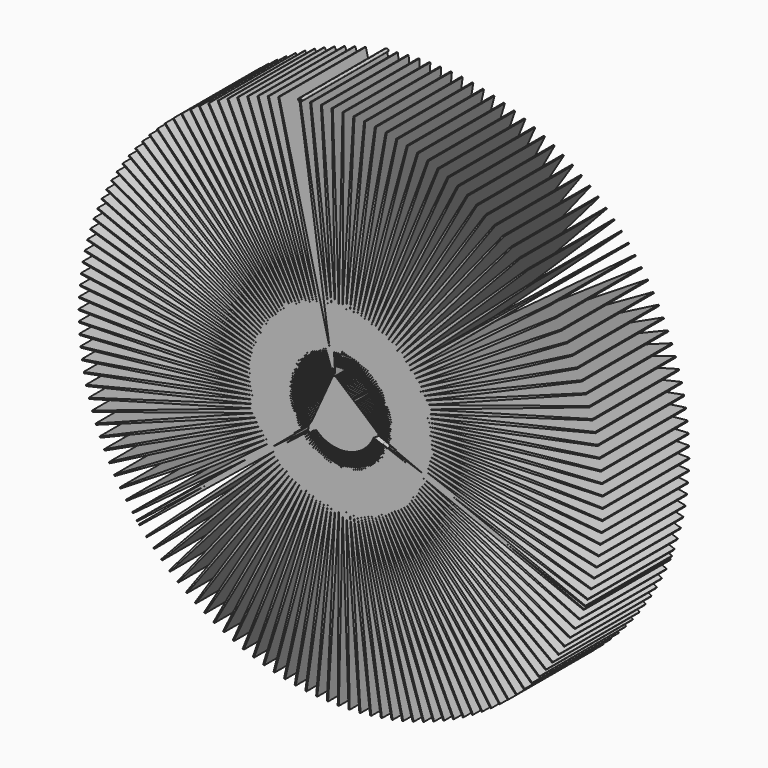
from build123d import *

# Parameters (mm, degrees)
F1_DEPTH = 25.4
F2_DEPTH = 25.4


with BuildPart() as f1:
    # F0 (on Front) → F1 (new body)
    with BuildSketch(Plane.XZ):
        Polygon((12.0425133313, 0.1286384218), (8.4582358292, 0.0040785031), (12.0375420948, -0.3691280198), (20.9257046857, -0.4277816267), align=None)
        Polygon((12.0269101358, 0.6261850868), (8.4508419081, 0.3536113969), (12.0425133313, 0.1286384218), (20.9255071427, 0.4373380094), align=None)
        Polygon((12.0375420948, -0.3691280198), (8.4511789962, -0.3454613587), (12.0120049195, -0.8662638124), (20.8901510133, -1.2921704052), align=None)
        Polygon((20.9257046857, -0.4277816267), (12.0375420948, -0.3691280198), (20.8901510133, -1.2921704052), (61.3826874331, -3.234697374), (61.3997078478, -2.9629681274), align=None)
        Polygon((20.9255071427, 0.4373380094), (12.0425133313, 0.1286384218), (20.9257046857, -0.4277816267), (61.4639255729, -0.6952961834), (61.4697022439, -0.4230956911), align=None)
        Polygon((20.8895587217, 1.3017104609), (12.0269101358, 0.6261850868), (20.9255071427, 0.4373380094), (61.4401536269, 1.8452929091), (61.4346766849, 2.1174995972), align=None)
        Polygon((8.4290098654, 0.7025401516), (12.0269101358, 0.6261850868), (20.8895587217, 1.3017104609), (11.9907591661, 1.1226619251), align=None)
        Polygon((20.8901510133, -1.2921704052), (12.0120049195, -0.8662638124), (20.8189068683, -2.1543515321), (61.1965780015, -5.7685721383), (61.2248130808, -5.4977783825), align=None)
        Polygon((20.8189068683, -2.1543515321), (12.0120049195, -0.8662638124), (8.4296834657, -0.6944110056), (11.9659454353, -1.3619196077), align=None)
        Polygon((11.9907591661, 1.1226619251), (20.8895587217, 1.3017104609), (61.311412209, 4.3827293496), (61.2946910113, 4.6544771729), (20.8179208401, 2.1638589619), align=None)
        Polygon((60.9453167476, -8.0231957753), (20.8189068683, -2.1543515321), (11.9659454353, -1.3619196077), (20.7120939701, -3.0128519856), (60.905915243, -8.292591394), align=None)
        Polygon((8.3927770008, 1.0502686282), (11.9907591661, 1.1226619251), (20.8179208401, 2.1638589619), (11.9341221855, 1.6172207143), align=None)
        Polygon((20.7120939701, -3.0128519856), (11.9659454353, -1.3619196077), (8.3937859623, -1.042174263), (11.899442334, -1.8552485863), align=None)
        Polygon((11.9341221855, 1.6172207143), (20.8179208401, 2.1638589619), (61.0779212718, 6.9126779705), (61.0499843863, 7.1835026525), (20.71071589, 3.0223105461), align=None)
        Polygon((60.5616963632, -10.5349056728), (20.7120939701, -3.0128519856), (11.899442334, -1.8552485863), (20.5698948068, -3.866205032), (60.5111957499, -10.8024428964), align=None)
        Polygon((8.3422052174, 1.3962027385), (11.9341221855, 1.6172207143), (20.71071589, 3.0223105461), (11.8570959574, 2.1090165091), align=None)
        Polygon((20.5698948068, -3.866205032), (11.899442334, -1.8552485863), (8.3435478165, -1.3881569831), (11.8126092352, -2.3454079038), align=None)
        Polygon((11.8570959574, 2.1090165091), (20.71071589, 3.0223105461), (60.7400797308, 9.4308163971), (60.700974887, 9.7002552382), (20.5681270292, 3.8755985635), align=None)
        Polygon((60.0746073364, -13.0286168607), (20.5698948068, -3.866205032), (11.8126092352, -2.3454079038), (20.3925523233, -4.712952732), (60.0130938939, -13.2938386063), align=None)
        Polygon((8.2773809164, 1.7397514598), (11.8570959574, 2.1090165091), (20.5681270292, 3.8755985635), (11.7598120797, 2.5972090846), align=None)
        Polygon((20.3925523233, -4.712952732), (11.8126092352, -2.3454079038), (8.2790548592, -1.7317680603), (11.7055944916, -2.8315601312), align=None)
        Polygon((11.7598120797, 2.5972090846), (20.5681270292, 3.8755985635), (60.2984647823, 11.932842432), (60.2482587904, 12.2004351006), (20.3903978683, 4.7222651858), align=None)
        Polygon((59.4848818506, -15.5000688752), (20.3925523233, -4.712952732), (11.7055944916, -2.8315601312), (20.1803695062, -5.5516484313), (59.4124606738, -15.7625220159), align=None)
        Polygon((8.1984148489, 2.0803278449), (11.7598120797, 2.5972090846), (20.3903978683, 4.7222651858), (11.6424367603, 3.0809643718), align=None)
        Polygon((20.1803695062, -5.5516484313), (11.7055944916, -2.8315601312), (8.2004172755, -2.0724204409), (11.5785809362, -3.3128746857), align=None)
        Polygon((11.6424367603, 3.0809643718), (20.3903978683, 4.7222651858), (59.7538309183, 14.4144814058), (59.6926095543, 14.6797707243), (20.1778320548, 5.5608638972), align=None)
        Polygon((58.7935274421, -17.945039282), (20.1803695062, -5.5516484313), (11.5785809362, -3.3128746857), (19.9337088664, -6.3808592323), (58.7103222611, -18.2042754211), align=None)
        Polygon((8.1054419271, 2.4173500248), (11.6424367603, 3.0809643718), (20.1778320548, 5.5608638972), (11.505170533, 3.5594558832), align=None)
        Polygon((19.9337088664, -6.3808592323), (11.5785809362, -3.3128746857), (9.0091905089, -2.644143551), (13.3303945996, -4.3674360381), align=None)
        Polygon((11.505170533, 3.5594558832), (20.1778320548, 5.5608638972), (59.1071086365, 16.8714934799), (59.0349764961, 17.134026206), (19.9307927536, 6.3899619659), align=None)
        Polygon((58.0017252782, -20.3593508903), (19.9337088664, -6.3808592323), (13.3303945996, -4.3674360381), (26.1031540688, -9.4612015654), (57.9078782478, -20.6149271271), align=None)
        Polygon((7.9986209938, 2.7502422027), (11.505170533, 3.5594558832), (19.9307927536, 6.3899619659), (11.3482479149, 4.0318661239), align=None)
        Polygon((26.1031540688, -9.4612015654), (13.3303945996, -4.3674360381), (11.4317855694, -3.7885292493), (19.6529918193, -7.1991684424), align=None)
        Polygon((11.3482479149, 4.0318661239), (19.9307927536, 6.3899619659), (58.3594028511, 19.2996808905), (58.2764831708, 19.5590084913), (19.6497020274, 7.2081428918), align=None)
        Polygon((57.4187139057, -21.949819984), (26.1031540688, -9.4612015654), (19.6529918193, -7.1991684424), (38.4148385654, -14.9826843771), (57.3178602732, -22.2027132871), align=None)
        Polygon((7.8781345507, 3.078435638), (11.3482479149, 4.0318661239), (19.6497020274, 7.2081428918), (11.1719370055, 4.4973879889), align=None)
        Polygon((38.4148385654, -14.9826843771), (19.6529918193, -7.1991684424), (11.2654591888, -4.2577111742), (15.5853834316, -6.2629501138), align=None)
        Polygon((11.1719370055, 4.4973879889), (19.6497020274, 7.2081428918), (57.5119910049, 21.6948951199), (57.4184254516, 21.9505745387), (19.3350401148, 8.0140088265), align=None)
        Polygon((57.1108281396, -22.738878889), (38.4148385654, -14.9826843771), (15.5853834316, -6.2629501138), (19.3386979654, -8.005177994), (57.0064995958, -22.9903585759), align=None)
        Polygon((7.7441884469, 3.4013696176), (11.1719370055, 4.4973879889), (19.3350401148, 8.0140088265), (10.9765390292, 4.955226142), align=None)
        Polygon((19.3386979654, -8.005177994), (15.5853834316, -6.2629501138), (9.7498261097, -4.034052892), (11.0798859602, -4.719618871), align=None)
        Polygon((10.9765390292, 4.955226142), (19.3350401148, 8.0140088265), (56.5663208868, 24.053043985), (56.4622693157, 24.3046383977), (18.9873446106, 8.8061829615), align=None)
        Polygon((56.1223581091, -25.0795578947), (19.3386979654, -8.005177994), (11.0798859602, -4.719618871), (18.9913642704, -8.7975108333), (56.0077262955, -25.3265113827), align=None)
        Polygon((7.597011527, 3.7184924143), (10.9765390292, 4.955226142), (18.9873446106, 8.8061829615), (10.7623878201, 5.4045983743), align=None)
        Polygon((18.9913642704, -8.7975108333), (11.0798859602, -4.719618871), (7.747465079, -3.3938996488), (10.8753829322, -5.1734631782), align=None)
        Polygon((10.7623878201, 5.4045983743), (18.9873446106, 8.8061829615), (55.5240081583, 26.3700986279), (55.4096483398, 26.6171781897), (18.6072095466, 9.5833118806), align=None)
        Polygon((55.0380039712, -27.3773888963), (18.9913642704, -8.7975108333), (10.8753829322, -5.1734631782), (18.6115841481, -9.5748132729), (54.9132647344, -27.6193942697), align=None)
        Polygon((7.4368552403, 4.029262229), (10.7623878201, 5.4045983743), (18.6072095466, 9.5833118806), (10.5298492519, 5.844736941), align=None)
        Polygon((18.6115841481, -9.5748132729), (10.8753829322, -5.1734631782), (7.6005940563, -3.7111642334), (10.6522994949, -5.6184687103), align=None)
        Polygon((10.5298492519, 5.844736941), (18.6072095466, 9.5833118806), (54.3868335933, 28.6421003997), (54.2623609092, 28.8842429792), (18.1952843772, 10.3440678722), align=None)
        Polygon((53.8596183268, -29.6284460883), (18.6115841481, -9.5748132729), (10.6522994949, -5.6184687103), (18.2000064465, -10.3357573046), (53.7249847816, -29.8650898848), align=None)
        Polygon((7.2639932113, 4.3331481169), (10.5298492519, 5.844736941), (18.1952843772, 10.3440678722), (10.2793206129, 6.2748898727), align=None)
        Polygon((18.2000064465, -10.3357573046), (10.6522994949, -5.6184687103), (7.4407375462, -4.0220883561), (10.4110167827, -6.0538751828), align=None)
        Polygon((10.2793206129, 6.2748898727), (18.1952843772, 10.3440678722), (53.1567400354, 30.8651676234), (53.0223671452, 31.1019595242), (17.7522728697, 11.0871511973), align=None)
        Polygon((52.589214428, -31.8288835771), (18.2000064465, -10.3357573046), (10.4110167827, -6.0538751828), (17.7573343392, -11.0790428683), (52.4449165935, -32.0597614949), align=None)
        Polygon((7.0787207717, 4.6296308938), (10.2793206129, 6.2748898727), (17.7522728697, 11.0871511973), (10.0112299271, 6.6943222603), align=None)
        Polygon((17.7573343392, -11.0790428683), (10.4110167827, -6.0538751828), (7.2681686608, -4.3261408084), (10.1519470229, -6.4789387112), align=None)
        Polygon((10.0112299271, 6.6943222603), (17.7522728697, 11.0871511973), (51.8358290789, 33.0355022259), (51.6917855563, 33.266538893), (17.2789319018, 11.8112923106), align=None)
        Polygon((51.2289627384, -33.9749419523), (17.7573343392, -11.0790428683), (10.1519470229, -6.4789387112), (17.2843241241, -11.8034000732), (51.0752471452, -34.1996595402), align=None)
        Polygon((6.8813544563, 4.9182040241), (10.0112299271, 6.6943222603), (17.2789319018, 11.8112923106), (9.7260352229, 7.1023175106), align=None)
        Polygon((17.2843241241, -11.8034000732), (10.1519470229, -6.4789387112), (7.0831822312, -4.6228021216), (9.8755328319, -6.8929330814), align=None)
        Polygon((9.7260352229, 7.1023175106), (17.2789319018, 11.8112923106), (50.4263574779, 35.1493962271), (50.272889419, 35.3742829381), (16.7760701686, 12.5152540291), align=None)
        Polygon((49.7811872254, -36.0629547091), (17.2843241241, -11.8034000732), (9.8755328319, -6.8929330814), (16.7817839311, -12.507591367), (49.6183164939, -36.2811280409), align=None)
        Polygon((6.6722314624, 5.1983744853), (9.7260352229, 7.1023175106), (16.7760701686, 12.5152540291), (9.4242237507, 7.4981785705), align=None)
        Polygon((16.7817839311, -12.507591367), (9.8755328319, -6.8929330814), (6.8860943036, -4.911565455), (9.5822464587, -7.2951509911), align=None)
        Polygon((9.4242237507, 7.4981785705), (16.7760701686, 12.5152540291), (48.930733291, 37.2032380744), (48.7681028933, 37.4215906143), (16.2445468008, 13.197833646), align=None)
        Polygon((48.2483613891, -38.0893545126), (16.7817839311, -12.507591367), (9.5822464587, -7.2951509911), (16.2505723417, -13.1904136508), (48.0766137812, -38.300610843), align=None)
        Polygon((6.4517090729, 5.4696636108), (9.4242237507, 7.4981785705), (16.2445468008, 13.197833646), (9.1063111502, 7.8812291182), align=None)
        Polygon((16.2505723417, -13.1904136508), (9.5822464587, -7.2951509911), (6.6772415993, -5.1919374612), (9.2725889782, -7.6849052577), align=None)
        Polygon((9.1063111502, 7.8812291182), (16.2445468008, 13.197833646), (47.3515117671, 39.1935188135), (47.179996882, 39.4049641306), (15.6852698974, 13.8578649856), align=None)
        Polygon((46.6331040366, -40.050679293), (16.2505723417, -13.1904136508), (9.2725889782, -7.6849052577), (15.6915969222, -13.8507003341), (46.4527729803, -40.2546576939), align=None)
        Polygon((6.2201640466, 5.7316079078), (9.1063111502, 7.8812291182), (15.6852698974, 13.8578649856), (8.7728405699, 8.2508147181), align=None)
        Polygon((15.6915969222, -13.8507003341), (9.2725889782, -7.6849052577), (6.4569809398, -5.4634391293), (8.9470894349, -8.0615299926), align=None)
        Polygon((8.7728405699, 8.2508147181), (15.6852698974, 13.8578649856), (45.6913909796, 41.1168380832), (45.5112846374, 41.3210149267), (15.0991949735, 14.4942203952), align=None)
        Polygon((44.9381748082, -41.9435781595), (15.6915969222, -13.8507003341), (8.9470894349, -8.0615299926), (15.1058126725, -14.4873233282), (44.749568396, -42.1399301374), align=None)
        Polygon((5.9779919745, 5.9837598489), (8.7728405699, 8.2508147181), (15.0991949735, 14.4942203952), (8.4243817387, 8.6063039395), align=None)
        Polygon((15.1058126725, -14.4873233282), (8.9470894349, -8.0615299926), (6.2256886367, -5.7256066033), (8.6063039395, -8.4243817387), align=None)
        Polygon((8.4243817387, 8.6063039395), (15.0991949735, 14.4942203952), (43.9532072171, 42.9699099248), (43.7648171264, 43.1664694619), (14.4873233283, 15.1058126725), align=None)
        Polygon((43.1664694619, -43.7648171264), (15.1058126725, -14.4873233282), (8.6063039395, -8.4243817387), (14.4942203952, -15.0991949735), (42.9699099248, -43.9532072171), align=None)
        Polygon((5.7256066033, 6.2256886367), (8.4243817387, 8.6063039395), (14.4873233283, 15.1058126725), (8.0615299926, 8.9470894349), align=None)
        Polygon((14.4942203952, -15.0991949735), (8.6063039395, -8.4243817387), (5.9837598489, -5.9779919745), (8.2508147181, -8.7728405699), align=None)
        Polygon((8.0615299926, 8.9470894349), (14.4873233283, 15.1058126725), (42.1399301374, 44.749568396), (41.9435781595, 44.9381748082), (13.8507003341, 15.6915969222), align=None)
        Polygon((41.3210149267, -45.5112846374), (14.4942203952, -15.0991949735), (8.2508147181, -8.7728405699), (13.8578649856, -15.6852698974), (41.1168380832, -45.6913909796), align=None)
        Polygon((5.4634391293, 6.4569809398), (8.0615299926, 8.9470894349), (13.8507003341, 15.6915969222), (7.6849052577, 9.2725889782), align=None)
        Polygon((13.8578649856, -15.6852698974), (8.2508147181, -8.7728405699), (5.7316079078, -6.2201640466), (7.8812291182, -9.1063111502), align=None)
        Polygon((7.6849052577, 9.2725889782), (13.8507003341, 15.6915969222), (40.2546576939, 46.4527729803), (40.050679293, 46.6331040366), (13.1904136508, 16.2505723417), align=None)
        Polygon((39.4049641306, -47.179996882), (13.8578649856, -15.6852698974), (7.8812291182, -9.1063111502), (13.197833646, -16.2445468008), (39.1935188135, -47.3515117671), align=None)
        Polygon((5.1919374612, 6.6772415993), (7.6849052577, 9.2725889782), (13.1904136508, 16.2505723417), (7.2951509911, 9.5822464587), align=None)
        Polygon((13.197833646, -16.2445468008), (7.8812291182, -9.1063111502), (5.4696636108, -6.4517090729), (7.4981785705, -9.4242237507), align=None)
        Polygon((7.2951509911, 9.5822464587), (13.1904136508, 16.2505723417), (38.300610843, 48.0766137812), (38.0893545126, 48.2483613891), (12.507591367, 16.7817839311), align=None)
        Polygon((37.4215906143, -48.7681028933), (13.197833646, -16.2445468008), (7.4981785705, -9.4242237507), (12.5152540291, -16.7760701686), (37.2032380744, -48.930733291), align=None)
        Polygon((4.911565455, 6.8860943036), (7.2951509911, 9.5822464587), (12.507591367, 16.7817839311), (6.8929330814, 9.8755328319), align=None)
        Polygon((12.5152540291, -16.7760701686), (7.4981785705, -9.4242237507), (5.1983744853, -6.6722314624), (7.1023175106, -9.7260352229), align=None)
        Polygon((6.8929330814, 9.8755328319), (12.507591367, 16.7817839311), (36.2811280409, 49.6183164939), (36.0629547091, 49.7811872254), (11.8034000732, 17.2843241241), align=None)
        Polygon((35.3742829381, -50.272889419), (12.5152540291, -16.7760701686), (7.1023175106, -9.7260352229), (11.8112923106, -17.2789319018), (35.1493962271, -50.4263574779), align=None)
        Polygon((4.6228021216, 7.0831822312), (6.8929330814, 9.8755328319), (11.8034000732, 17.2843241241), (6.4789387112, 10.1519470229), align=None)
        Polygon((11.8112923106, -17.2789319018), (7.1023175106, -9.7260352229), (4.9182040241, -6.8813544563), (6.6943222603, -10.0112299271), align=None)
        Polygon((6.4789387112, 10.1519470229), (11.8034000732, 17.2843241241), (34.1996595402, 51.0752471452), (33.9749419523, 51.2289627384), (11.0790428683, 17.7573343392), align=None)
        Polygon((33.266538893, -51.6917855563), (11.8112923106, -17.2789319018), (6.6943222603, -10.0112299271), (11.0871511973, -17.7522728697), (33.0355022259, -51.8358290789), align=None)
        Polygon((4.3261408084, 7.2681686608), (6.4789387112, 10.1519470229), (11.0790428683, 17.7573343392), (6.0538751828, 10.4110167827), align=None)
        Polygon((11.0871511973, -17.7522728697), (6.6943222603, -10.0112299271), (4.6296308938, -7.0787207717), (6.2748898727, -10.2793206129), align=None)
        Polygon((6.0538751828, 10.4110167827), (11.0790428683, 17.7573343392), (32.0597614949, 52.4449165935), (31.8288835771, 52.589214428), (10.3357573046, 18.2000064465), align=None)
        Polygon((31.1019595242, -53.0223671452), (11.0871511973, -17.7522728697), (6.2748898727, -10.2793206129), (10.3440678722, -18.1952843772), (30.8651676234, -53.1567400354), align=None)
        Polygon((4.0220883561, 7.4407375462), (6.0538751828, 10.4110167827), (10.3357573046, 18.2000064465), (5.6184687103, 10.6522994949), align=None)
        Polygon((10.3440678722, -18.1952843772), (6.2748898727, -10.2793206129), (4.3331481169, -7.2639932113), (5.844736941, -10.5298492519), align=None)
        Polygon((5.6184687103, 10.6522994949), (10.3357573046, 18.2000064465), (29.8650898848, 53.7249847816), (29.6284460883, 53.8596183268), (9.5748132729, 18.6115841481), align=None)
        Polygon((28.8842429792, -54.2623609092), (10.3440678722, -18.1952843772), (5.844736941, -10.5298492519), (9.5833118806, -18.6072095466), (28.6421003997, -54.3868335933), align=None)
        Polygon((3.7111642334, 7.6005940563), (5.6184687103, 10.6522994949), (9.5748132729, 18.6115841481), (5.1734631782, 10.8753829322), align=None)
        Polygon((9.5833118806, -18.6072095466), (5.844736941, -10.5298492519), (4.029262229, -7.4368552403), (5.4045983743, -10.7623878201), align=None)
        Polygon((5.1734631782, 10.8753829322), (9.5748132729, 18.6115841481), (27.6193942697, 54.9132647344), (27.3773888963, 55.0380039712), (8.7975108333, 18.9913642704), align=None)
        Polygon((26.6171781897, -55.4096483398), (9.5833118806, -18.6072095466), (5.4045983743, -10.7623878201), (8.8061829615, -18.9873446106), (26.3700986279, -55.5240081583), align=None)
        Polygon((3.3938996488, 7.747465079), (5.1734631782, 10.8753829322), (8.7975108333, 18.9913642704), (4.719618871, 11.0798859602), align=None)
        Polygon((8.8061829615, -18.9873446106), (5.4045983743, -10.7623878201), (3.7184924143, -7.597011527), (4.955226142, -10.9765390292), align=None)
        Polygon((4.719618871, 11.0798859602), (8.7975108333, 18.9913642704), (25.3265113827, 56.0077262955), (25.0795578947, 56.1223581091), (8.005177994, 19.3386979654), align=None)
        Polygon((24.3046383977, -56.4622693157), (8.8061829615, -18.9873446106), (4.955226142, -10.9765390292), (8.0140088265, -19.3350401148), (24.053043985, -56.5663208868), align=None)
        Polygon((3.0708366436, 7.8810996875), (4.719618871, 11.0798859602), (8.005177994, 19.3386979654), (4.2577111742, 11.2654591888), align=None)
        Polygon((8.0140088265, -19.3350401148), (4.955226142, -10.9765390292), (3.4013696176, -7.7441884469), (4.4973879889, -11.1719370055), align=None)
        Polygon((4.2577111742, 11.2654591888), (8.005177994, 19.3386979654), (22.9903585759, 57.0064995958), (22.738878889, 57.1108281396), (7.1991684424, 19.6529918193), align=None)
        Polygon((21.9505745387, -57.4184254516), (8.0140088265, -19.3350401148), (4.4973879889, -11.1719370055), (7.2081428918, -19.6497020274), (21.6948951199, -57.5119910049), align=None)
        Polygon((2.7425271656, 8.0012695694), (4.2577111742, 11.2654591888), (7.1991684424, 19.6529918193), (3.7885292493, 11.4317855694), align=None)
        Polygon((7.2081428918, -19.6497020274), (4.4973879889, -11.1719370055), (3.078435638, -7.8781345507), (4.0318661239, -11.3482479149), align=None)
        Polygon((3.7885292493, 11.4317855694), (7.1991684424, 19.6529918193), (20.6149271271, 57.9078782478), (20.3593508903, 58.0017252782), (6.3808592323, 19.9337088664), align=None)
        Polygon((19.5590084913, -58.2764831708), (7.2081428918, -19.6497020274), (4.0318661239, -11.3482479149), (6.3899619659, -19.9307927536), (19.2996808905, -58.3594028511), align=None)
        Polygon((2.4095321258, 8.1077694165), (3.7885292493, 11.4317855694), (6.3808592323, 19.9337088664), (3.3128746857, 11.5785809362), align=None)
        Polygon((6.3899619659, -19.9307927536), (4.0318661239, -11.3482479149), (2.7502422027, -7.9986209938), (3.5594558832, -11.505170533), align=None)
        Polygon((3.3128746857, 11.5785809362), (6.3808592323, 19.9337088664), (18.2042754211, 58.7103222611), (17.945039282, 58.7935274421), (5.5516484313, 20.1803695062), align=None)
        Polygon((17.134026206, -59.0349764961), (6.3899619659, -19.9307927536), (3.5594558832, -11.505170533), (5.5608638972, -20.1778320548), (16.8714934799, -59.1071086365), align=None)
        Polygon((2.0724204409, 8.2004172755), (3.3128746857, 11.5785809362), (5.5516484313, 20.1803695062), (2.8315601312, 11.7055944916), align=None)
        Polygon((5.5608638972, -20.1778320548), (3.5594558832, -11.505170533), (2.4173500248, -8.1054419271), (3.0809643718, -11.6424367603), align=None)
        Polygon((2.8315601312, 11.7055944916), (5.5516484313, 20.1803695062), (15.7625220159, 59.4124606738), (15.5000688752, 59.4848818506), (4.712952732, 20.3925523233), align=None)
        Polygon((14.6797707243, -59.6926095543), (5.5608638972, -20.1778320548), (3.0809643718, -11.6424367603), (4.7222651858, -20.3903978683), (14.4144814058, -59.7538309183), align=None)
        Polygon((1.7317680603, 8.2790548592), (2.8315601312, 11.7055944916), (4.712952732, 20.3925523233), (2.3454079038, 11.8126092352), align=None)
        Polygon((4.7222651858, -20.3903978683), (3.0809643718, -11.6424367603), (2.0803278449, -8.1984148489), (2.5972090846, -11.7598120797), align=None)
        Polygon((2.3454079038, 11.8126092352), (4.712952732, 20.3925523233), (13.2938386063, 60.0130938939), (13.0286168607, 60.0746073364), (3.866205032, 20.5698948068), align=None)
        Polygon((12.2004351006, -60.2482587904), (4.7222651858, -20.3903978683), (2.5972090846, -11.7598120797), (3.8755985635, -20.5681270292), (11.932842432, -60.2984647823), align=None)
        Polygon((1.3881569831, 8.3435478165), (2.3454079038, 11.8126092352), (3.866205032, 20.5698948068), (1.8552485863, 11.899442334), align=None)
        Polygon((3.8755985635, -20.5681270292), (2.5972090846, -11.7598120797), (1.7397514598, -8.2773809164), (2.1090165091, -11.8570959574), align=None)
        Polygon((1.8552485863, 11.899442334), (3.866205032, 20.5698948068), (10.8024428964, 60.5111957499), (10.5349056728, 60.5616963632), (3.0128519856, 20.7120939701), align=None)
        Polygon((9.7002552382, -60.700974887), (3.8755985635, -20.5681270292), (2.1090165091, -11.8570959574), (3.0223105461, -20.71071589), (9.4308163971, -60.7400797308), align=None)
        Polygon((1.042174263, 8.3937859623), (1.8552485863, 11.899442334), (3.0128519856, 20.7120939701), (1.3619196077, 11.9659454353), align=None)
        Polygon((3.0223105461, -20.71071589), (2.1090165091, -11.8570959574), (1.3962027385, -8.3422052174), (1.6172207143, -11.9341221855), align=None)
        Polygon((1.3619196077, 11.9659454353), (3.0128519856, 20.7120939701), (8.292591394, 60.905915243), (8.0231957753, 60.9453167476), (2.1543515321, 20.8189068683), align=None)
        Polygon((7.1835026525, -61.0499843863), (3.0223105461, -20.71071589), (1.6172207143, -11.9341221855), (2.1638589619, -20.8179208401), (6.9126779705, -61.0779212718), align=None)
        Polygon((0.6944110056, 8.4296834657), (1.3619196077, 11.9659454353), (2.1543515321, 20.8189068683), (0.8662638124, 12.0120049195), align=None)
        Polygon((2.1638589619, -20.8179208401), (1.6172207143, -11.9341221855), (1.0502686282, -8.3927770008), (1.1226619251, -11.9907591661), align=None)
        Polygon((0.8662638124, 12.0120049195), (2.1543515321, 20.8189068683), (5.7685721383, 61.1965780015), (5.4977783825, 61.2248130808), (1.2921704052, 20.8901510133), align=None)
        Polygon((4.6544771729, -61.2946910113), (2.1638589619, -20.8179208401), (1.1226619251, -11.9907591661), (1.3017104609, -20.8895587217), (4.3827293496, -61.311412209), align=None)
        Polygon((0.3454613587, 8.4511789962), (0.8662638124, 12.0120049195), (1.2921704052, 20.8901510133), (0.3691280198, 12.0375420948), align=None)
        Polygon((1.3017104609, -20.8895587217), (1.1226619251, -11.9907591661), (0.7025401516, -8.4290098654), (0.6261850868, -12.0269101358), align=None)
        Polygon((0.3691280198, 12.0375420948), (1.2921704052, 20.8901510133), (3.234697374, 61.3826874331), (2.9629681274, 61.3997078478), (0.4277816267, 20.9257046857), align=None)
        Polygon((2.1174995972, -61.4346766849), (1.3017104609, -20.8895587217), (0.6261850868, -12.0269101358), (0.4373380094, -20.9255071427), (1.8452929091, -61.4401536269), align=None)
        Polygon((-0.0040785031, 8.4582358292), (0.3691280198, 12.0375420948), (0.4277816267, 20.9257046857), (-0.1286384218, 12.0425133313), align=None)
        Polygon((0.4373380094, -20.9255071427), (0.6261850868, -12.0269101358), (0.3536113969, -8.4508419081), (0.1286384218, -12.0425133313), align=None)
        Polygon((-0.1286384218, 12.0425133313), (0.4277816267, 20.9257046857), (0.6952961834, 61.4639255729), (0.4230956911, 61.4697022439), (-0.4373380094, 20.9255071427), align=None)
        Polygon((-0.4230956911, -61.4697022439), (0.4373380094, -20.9255071427), (0.1286384218, -12.0425133313), (-0.4277816267, -20.9257046857), (-0.6952961834, -61.4639255729), align=None)
        Polygon((-0.3536113969, 8.4508419081), (-0.1286384218, 12.0425133313), (-0.4373380094, 20.9255071427), (-0.6261850868, 12.0269101358), align=None)
        Polygon((-0.4277816267, -20.9257046857), (0.1286384218, -12.0425133313), (0.0040785031, -8.4582358292), (-0.3691280198, -12.0375420948), align=None)
        Polygon((-0.6261850868, 12.0269101358), (-0.4373380094, 20.9255071427), (-1.8452929091, 61.4401536269), (-2.1174995972, 61.4346766849), (-1.3017104609, 20.8895587217), align=None)
        Polygon((-2.9629681274, -61.3997078478), (-0.4277816267, -20.9257046857), (-0.3691280198, -12.0375420948), (-1.2921704052, -20.8901510133), (-3.234697374, -61.3826874331), align=None)
        Polygon((-0.7025401516, 8.4290098654), (-0.6261850868, 12.0269101358), (-1.3017104609, 20.8895587217), (-1.1226619251, 11.9907591661), align=None)
        Polygon((-1.2921704052, -20.8901510133), (-0.3691280198, -12.0375420948), (-0.3454613587, -8.4511789962), (-0.8662638124, -12.0120049195), align=None)
        Polygon((-1.1226619251, 11.9907591661), (-1.3017104609, 20.8895587217), (-4.3827293496, 61.311412209), (-4.6544771729, 61.2946910113), (-2.1638589619, 20.8179208401), align=None)
        Polygon((-5.4977783825, -61.2248130808), (-1.2921704052, -20.8901510133), (-0.8662638124, -12.0120049195), (-2.1543515321, -20.8189068683), (-5.7685721383, -61.1965780015), align=None)
        Polygon((-1.0502686282, 8.3927770008), (-1.1226619251, 11.9907591661), (-2.1638589619, 20.8179208401), (-1.6172207143, 11.9341221855), align=None)
        Polygon((-2.1543515321, -20.8189068683), (-0.8662638124, -12.0120049195), (-0.6944110056, -8.4296834657), (-1.3619196077, -11.9659454353), align=None)
        Polygon((-1.6172207143, 11.9341221855), (-2.1638589619, 20.8179208401), (-6.9126779705, 61.0779212718), (-7.1835026525, 61.0499843863), (-3.0223105461, 20.71071589), align=None)
        Polygon((-8.0231957753, -60.9453167476), (-2.1543515321, -20.8189068683), (-1.3619196077, -11.9659454353), (-3.0128519856, -20.7120939701), (-8.292591394, -60.905915243), align=None)
        Polygon((-1.2764281614, 6.395665195), (-1.6172207143, 11.9341221855), (-3.0223105461, 20.71071589), (-1.7397514598, 8.2773809164), align=None)
        Polygon((-3.0128519856, -20.7120939701), (-1.3619196077, -11.9659454353), (-1.042174263, -8.3937859623), (-1.8552485863, -11.899442334), align=None)
        with BuildLine():
            Line((-1.7397514598, 8.2773809164), (-3.0223105461, 20.71071589))
            Line((-3.0223105461, 20.71071589), (-9.3816127043, 60.4327393671))
            ThreePointArc((-9.3816127043, 60.4327393671), (-9.4569735765, 60.4297474622), (-9.5308850368, 60.4447577446))
            ThreePointArc((-9.5308850368, 60.4447577446), (-9.5908771837, 60.4139732661), (-9.6561411994, 60.397021863))
            Line((-9.6561411994, 60.397021863), (-2.5972090846, 11.7598120797))
            Line((-2.5972090846, 11.7598120797), (-1.7397514598, 8.2773809164))
        make_face()
        Polygon((-10.5349056728, -60.5616963632), (-3.0128519856, -20.7120939701), (-1.8552485863, -11.899442334), (-3.866205032, -20.5698948068), (-10.8024428964, -60.5111957499), align=None)
        Polygon((-1.5396384828, 6.3374533907), (-1.7397514598, 8.2773809164), (-2.5972090846, 11.7598120797), (-2.0803278449, 8.1984148489), align=None)
        with BuildLine():
            ThreePointArc((-9.5308850368, 60.4447577446), (-9.4569735765, 60.4297474622), (-9.3816127043, 60.4327393671))
            Line((-9.3816127043, 60.4327393671), (-9.408965222, 60.6035910299))
            ThreePointArc((-9.408965222, 60.6035910299), (-9.4566182907, 60.5139601094), (-9.5308850368, 60.4447577446))
        make_face()
        with BuildLine():
            Line((-9.408965222, 60.6035910299), (-9.3816127043, 60.4327393671))
            ThreePointArc((-9.3816127043, 60.4327393671), (-9.1919365401, 60.5394533767), (-9.1167431918, 60.7436858118))
            ThreePointArc((-9.1167431918, 60.7436858118), (-9.2897639484, 61.0248460122), (-9.6187276022, 60.9970943456))
            ThreePointArc((-9.6187276022, 60.9970943456), (-9.4559463257, 60.8871109782), (-9.3931176645, 60.700974887))
            ThreePointArc((-9.3931176645, 60.700974887), (-9.3971054419, 60.6516424415), (-9.408965222, 60.6035910299))
        make_face()
        Polygon((-3.866205032, -20.5698948068), (-1.8552485863, -11.899442334), (-1.3881569831, -8.3435478165), (-2.3454079038, -11.8126092352), align=None)
        Polygon((-2.0803278449, 8.1984148489), (-2.5972090846, 11.7598120797), (-14.4144814058, 59.7538309183), (-14.6797707243, 59.6926095543), (-5.5608638972, 20.1778320548), align=None)
        with BuildLine():
            Line((-9.4308163971, 60.7400797308), (-9.408965222, 60.6035910299))
            ThreePointArc((-9.408965222, 60.6035910299), (-9.3971054419, 60.6516424415), (-9.3931176645, 60.700974887))
            ThreePointArc((-9.3931176645, 60.700974887), (-9.4559463257, 60.8871109782), (-9.6187276022, 60.9970943456))
            ThreePointArc((-9.6187276022, 60.9970943456), (-9.7439555471, 60.7848080468), (-9.6779573261, 60.5473385843))
            Line((-9.6779573261, 60.5473385843), (-9.7002552382, 60.700974887))
            Line((-9.7002552382, 60.700974887), (-9.4308163971, 60.7400797308))
        make_face()
        with BuildLine():
            ThreePointArc((-9.6561411994, 60.397021863), (-9.5908771837, 60.4139732661), (-9.5308850368, 60.4447577446))
            ThreePointArc((-9.5308850368, 60.4447577446), (-9.6118756791, 60.4853604957), (-9.6779573261, 60.5473385843))
            Line((-9.6779573261, 60.5473385843), (-9.6561411994, 60.397021863))
        make_face()
        Polygon((-13.0286168607, -60.0746073364), (-3.866205032, -20.5698948068), (-2.3454079038, -11.8126092352), (-4.712952732, -20.3925523233), (-13.2938386063, -60.0130938939), align=None)
        Polygon((-1.8002183578, 6.2684141537), (-2.0803278449, 8.1984148489), (-5.5608638972, 20.1778320548), (-3.5594558832, 11.505170533), align=None)
        with BuildLine():
            ThreePointArc((-9.8120783988, 60.9870326958), (-9.9971968604, 60.6224945568), (-9.6561411994, 60.397021863))
            Line((-9.6561411994, 60.397021863), (-9.6779573261, 60.5473385843))
            ThreePointArc((-9.6779573261, 60.5473385843), (-9.7439555471, 60.7848080468), (-9.6187276022, 60.9970943456))
            ThreePointArc((-9.6187276022, 60.9970943456), (-9.7162165634, 61.0076974413), (-9.8120783988, 60.9870326958))
        make_face()
        Polygon((-4.712952732, -20.3925523233), (-2.3454079038, -11.8126092352), (-1.7317680603, -8.2790548592), (-2.8315601312, -11.7055944916), align=None)
        Polygon((-3.5594558832, 11.505170533), (-5.5608638972, 20.1778320548), (-16.8714934799, 59.1071086365), (-17.134026206, 59.0349764961), (-6.3899619659, 19.9307927536), align=None)
        Polygon((-15.5000688752, -59.4848818506), (-4.712952732, -20.3925523233), (-2.8315601312, -11.7055944916), (-5.5516484313, -20.1803695062), (-15.7625220159, -59.4124606738), align=None)
        Polygon((-2.7502422027, 7.9986209938), (-3.5594558832, 11.505170533), (-6.3899619659, 19.9307927536), (-4.0318661239, 11.3482479149), align=None)
        Polygon((-5.5516484313, -20.1803695062), (-2.8315601312, -11.7055944916), (-2.0724204409, -8.2004172755), (-3.3128746857, -11.5785809362), align=None)
        Polygon((-4.0318661239, 11.3482479149), (-6.3899619659, 19.9307927536), (-19.2996808905, 58.3594028511), (-19.5590084913, 58.2764831708), (-7.2081428918, 19.6497020274), align=None)
        Polygon((-17.945039282, -58.7935274421), (-5.5516484313, -20.1803695062), (-3.3128746857, -11.5785809362), (-6.3808592323, -19.9337088664), (-18.2042754211, -58.7103222611), align=None)
        Polygon((-3.078435638, 7.8781345507), (-4.0318661239, 11.3482479149), (-7.2081428918, 19.6497020274), (-4.4973879889, 11.1719370055), align=None)
        Polygon((-6.3808592323, -19.9337088664), (-3.3128746857, -11.5785809362), (-2.4095321258, -8.1077694165), (-3.7885292493, -11.4317855694), align=None)
        Polygon((-4.4973879889, 11.1719370055), (-7.2081428918, 19.6497020274), (-21.6948951199, 57.5119910049), (-21.9505745387, 57.4184254516), (-8.0140088265, 19.3350401148), align=None)
        Polygon((-20.3593508903, -58.0017252782), (-6.3808592323, -19.9337088664), (-3.7885292493, -11.4317855694), (-7.1991684424, -19.6529918193), (-20.6149271271, -57.9078782478), align=None)
        Polygon((-3.4013696176, 7.7441884469), (-4.4973879889, 11.1719370055), (-8.0140088265, 19.3350401148), (-4.955226142, 10.9765390292), align=None)
        Polygon((-7.1991684424, -19.6529918193), (-3.7885292493, -11.4317855694), (-2.7425271656, -8.0012695694), (-4.2577111742, -11.2654591888), align=None)
        Polygon((-4.955226142, 10.9765390292), (-8.0140088265, 19.3350401148), (-24.053043985, 56.5663208868), (-24.3046383977, 56.4622693157), (-8.8061829615, 18.9873446106), align=None)
        Polygon((-22.738878889, -57.1108281396), (-7.1991684424, -19.6529918193), (-4.2577111742, -11.2654591888), (-8.005177994, -19.3386979654), (-22.9903585759, -57.0064995958), align=None)
        Polygon((-3.7184924143, 7.597011527), (-4.955226142, 10.9765390292), (-8.8061829615, 18.9873446106), (-5.4045983743, 10.7623878201), align=None)
        Polygon((-8.005177994, -19.3386979654), (-4.2577111742, -11.2654591888), (-3.0708366436, -7.8810996875), (-4.719618871, -11.0798859602), align=None)
        Polygon((-5.4045983743, 10.7623878201), (-8.8061829615, 18.9873446106), (-26.3700986279, 55.5240081583), (-26.6171781897, 55.4096483398), (-9.5833118806, 18.6072095466), align=None)
        Polygon((-25.0795578947, -56.1223581091), (-8.005177994, -19.3386979654), (-4.719618871, -11.0798859602), (-8.7975108333, -18.9913642704), (-25.3265113827, -56.0077262955), align=None)
        Polygon((-4.029262229, 7.4368552403), (-5.4045983743, 10.7623878201), (-9.5833118806, 18.6072095466), (-5.844736941, 10.5298492519), align=None)
        Polygon((-8.7975108333, -18.9913642704), (-4.719618871, -11.0798859602), (-3.3938996488, -7.747465079), (-5.1734631782, -10.8753829322), align=None)
        Polygon((-5.844736941, 10.5298492519), (-9.5833118806, 18.6072095466), (-28.6421003997, 54.3868335933), (-28.8842429792, 54.2623609092), (-10.3440678722, 18.1952843772), align=None)
        Polygon((-27.3773888963, -55.0380039712), (-8.7975108333, -18.9913642704), (-5.1734631782, -10.8753829322), (-9.5748132729, -18.6115841481), (-27.6193942697, -54.9132647344), align=None)
        Polygon((-4.3331481169, 7.2639932113), (-5.844736941, 10.5298492519), (-10.3440678722, 18.1952843772), (-6.2748898727, 10.2793206129), align=None)
        Polygon((-9.5748132729, -18.6115841481), (-5.1734631782, -10.8753829322), (-3.7111642334, -7.6005940563), (-5.6184687103, -10.6522994949), align=None)
        Polygon((-6.2748898727, 10.2793206129), (-10.3440678722, 18.1952843772), (-30.8651676234, 53.1567400354), (-31.1019595242, 53.0223671452), (-11.0871511973, 17.7522728697), align=None)
        Polygon((-29.6284460883, -53.8596183268), (-9.5748132729, -18.6115841481), (-5.6184687103, -10.6522994949), (-10.3357573046, -18.2000064465), (-29.8650898848, -53.7249847816), align=None)
        Polygon((-4.6296308938, 7.0787207717), (-6.2748898727, 10.2793206129), (-11.0871511973, 17.7522728697), (-6.6943222603, 10.0112299271), align=None)
        Polygon((-10.3357573046, -18.2000064465), (-5.6184687103, -10.6522994949), (-4.0220883561, -7.4407375462), (-6.0538751828, -10.4110167827), align=None)
        Polygon((-6.6943222603, 10.0112299271), (-11.0871511973, 17.7522728697), (-33.0355022259, 51.8358290789), (-33.266538893, 51.6917855563), (-11.8112923106, 17.2789319018), align=None)
        Polygon((-31.8288835771, -52.589214428), (-10.3357573046, -18.2000064465), (-6.0538751828, -10.4110167827), (-11.0790428683, -17.7573343392), (-32.0597614949, -52.4449165935), align=None)
        Polygon((-4.9182040241, 6.8813544563), (-6.6943222603, 10.0112299271), (-11.8112923106, 17.2789319018), (-7.1023175106, 9.7260352229), align=None)
        Polygon((-11.0790428683, -17.7573343392), (-6.0538751828, -10.4110167827), (-4.3261408084, -7.2681686608), (-6.4789387112, -10.1519470229), align=None)
        Polygon((-7.1023175106, 9.7260352229), (-11.8112923106, 17.2789319018), (-35.1493962271, 50.4263574779), (-35.3742829381, 50.272889419), (-12.5152540291, 16.7760701686), align=None)
        Polygon((-33.9749419523, -51.2289627384), (-11.0790428683, -17.7573343392), (-6.4789387112, -10.1519470229), (-11.8034000732, -17.2843241241), (-34.1996595402, -51.0752471452), align=None)
        Polygon((-5.1983744853, 6.6722314624), (-7.1023175106, 9.7260352229), (-12.5152540291, 16.7760701686), (-7.4981785705, 9.4242237507), align=None)
        Polygon((-11.8034000732, -17.2843241241), (-6.4789387112, -10.1519470229), (-4.6228021216, -7.0831822312), (-6.8929330814, -9.8755328319), align=None)
        Polygon((-7.4981785705, 9.4242237507), (-12.5152540291, 16.7760701686), (-37.2032380744, 48.930733291), (-37.4215906143, 48.7681028933), (-13.197833646, 16.2445468008), align=None)
        Polygon((-36.0629547091, -49.7811872254), (-11.8034000732, -17.2843241241), (-6.8929330814, -9.8755328319), (-12.507591367, -16.7817839311), (-36.2811280409, -49.6183164939), align=None)
        Polygon((-5.4696636108, 6.4517090729), (-7.4981785705, 9.4242237507), (-13.197833646, 16.2445468008), (-7.8812291182, 9.1063111502), align=None)
        Polygon((-12.507591367, -16.7817839311), (-6.8929330814, -9.8755328319), (-4.911565455, -6.8860943036), (-7.2951509911, -9.5822464587), align=None)
        Polygon((-7.8812291182, 9.1063111502), (-13.197833646, 16.2445468008), (-39.1935188135, 47.3515117671), (-39.4049641306, 47.179996882), (-13.8578649856, 15.6852698974), align=None)
        Polygon((-38.0893545126, -48.2483613891), (-12.507591367, -16.7817839311), (-7.2951509911, -9.5822464587), (-13.1904136508, -16.2505723417), (-38.300610843, -48.0766137812), align=None)
        Polygon((-5.7316079078, 6.2201640466), (-7.8812291182, 9.1063111502), (-13.8578649856, 15.6852698974), (-8.2508147181, 8.7728405699), align=None)
        Polygon((-13.1904136508, -16.2505723417), (-7.2951509911, -9.5822464587), (-5.1919374612, -6.6772415993), (-7.6849052577, -9.2725889782), align=None)
        Polygon((-8.2508147181, 8.7728405699), (-13.8578649856, 15.6852698974), (-41.1168380832, 45.6913909796), (-41.3210149267, 45.5112846374), (-14.4942203952, 15.0991949735), align=None)
        Polygon((-40.050679293, -46.6331040366), (-13.1904136508, -16.2505723417), (-7.6849052577, -9.2725889782), (-13.8507003341, -15.6915969222), (-40.2546576939, -46.4527729803), align=None)
        Polygon((-5.9837598489, 5.9779919745), (-8.2508147181, 8.7728405699), (-14.4942203952, 15.0991949735), (-8.6063039395, 8.4243817387), align=None)
        Polygon((-13.8507003341, -15.6915969222), (-7.6849052577, -9.2725889782), (-5.4634391293, -6.4569809398), (-8.0615299926, -8.9470894349), align=None)
        Polygon((-8.6063039395, 8.4243817387), (-14.4942203952, 15.0991949735), (-42.9699099248, 43.9532072171), (-43.1664694619, 43.7648171264), (-15.1058126725, 14.4873233283), align=None)
        Polygon((-41.9435781595, -44.9381748082), (-13.8507003341, -15.6915969222), (-8.0615299926, -8.9470894349), (-14.4873233282, -15.1058126725), (-42.1399301374, -44.749568396), align=None)
        Polygon((-6.2256886367, 5.7256066033), (-8.6063039395, 8.4243817387), (-15.1058126725, 14.4873233283), (-8.9470894349, 8.0615299926), align=None)
        Polygon((-14.4873233282, -15.1058126725), (-8.0615299926, -8.9470894349), (-5.7256066033, -6.2256886367), (-8.4243817387, -8.6063039395), align=None)
        Polygon((-8.9470894349, 8.0615299926), (-15.1058126725, 14.4873233283), (-44.749568396, 42.1399301374), (-44.9381748082, 41.9435781595), (-15.6915969222, 13.8507003341), align=None)
        Polygon((-43.7648171264, -43.1664694619), (-14.4873233282, -15.1058126725), (-8.4243817387, -8.6063039395), (-15.0991949735, -14.4942203952), (-43.9532072171, -42.9699099248), align=None)
        Polygon((-6.4569809398, 5.4634391293), (-8.9470894349, 8.0615299926), (-15.6915969222, 13.8507003341), (-9.2725889782, 7.6849052577), align=None)
        Polygon((-15.0991949735, -14.4942203952), (-8.4243817387, -8.6063039395), (-5.9779919745, -5.9837598489), (-8.7728405699, -8.2508147181), align=None)
        Polygon((-9.2725889782, 7.6849052577), (-15.6915969222, 13.8507003341), (-46.4527729803, 40.2546576939), (-46.6331040366, 40.050679293), (-16.2505723417, 13.1904136508), align=None)
        Polygon((-45.5112846374, -41.3210149267), (-15.0991949735, -14.4942203952), (-8.7728405699, -8.2508147181), (-15.6852698974, -13.8578649856), (-45.6913909796, -41.1168380832), align=None)
        Polygon((-6.6772415993, 5.1919374612), (-9.2725889782, 7.6849052577), (-16.2505723417, 13.1904136508), (-9.5822464587, 7.2951509911), align=None)
        Polygon((-15.6852698974, -13.8578649856), (-8.7728405699, -8.2508147181), (-7.7107115752, -7.2026119504), (-12.6254643067, -11.0781935295), align=None)
        Polygon((-9.5822464587, 7.2951509911), (-16.2505723417, 13.1904136508), (-48.0766137812, 38.300610843), (-48.2483613891, 38.0893545126), (-16.7817839311, 12.507591367), align=None)
        Polygon((-47.179996882, -39.4049641306), (-15.6852698974, -13.8578649856), (-12.6254643067, -11.0781935295), (-31.8245832719, -26.2178670514), (-47.3515117671, -39.1935188135), align=None)
        Polygon((-6.8860943036, 4.911565455), (-9.5822464587, 7.2951509911), (-16.7817839311, 12.507591367), (-9.8755328319, 6.8929330814), align=None)
        Polygon((-31.8245832719, -26.2178670514), (-12.6254643067, -11.0781935295), (-9.1063111502, -7.8812291182), (-16.2445468008, -13.197833646), align=None)
        Polygon((-9.8755328319, 6.8929330814), (-16.7817839311, 12.507591367), (-49.6183164939, 36.2811280409), (-49.7811872254, 36.0629547091), (-17.2843241241, 11.8034000732), align=None)
        Polygon((-47.7184586675, -38.751154903), (-31.8245832719, -26.2178670514), (-16.2445468008, -13.197833646), (-21.729696, -17.2832085895), (-47.8870438762, -38.5373664437), align=None)
        Polygon((-7.0831822312, 4.6228021216), (-9.8755328319, 6.8929330814), (-17.2843241241, 11.8034000732), (-10.1519470229, 6.4789387112), align=None)
        Polygon((-21.729696, -17.2832085895), (-16.2445468008, -13.197833646), (-9.4242237507, -7.4981785705), (-11.0671176359, -8.619328568), align=None)
        Polygon((-10.1519470229, 6.4789387112), (-17.2843241241, 11.8034000732), (-51.0752471452, 34.1996595402), (-51.2289627384, 33.9749419523), (-17.7573343392, 11.0790428683), align=None)
        Polygon((-48.7681028933, -37.4215906143), (-21.729696, -17.2832085895), (-11.0671176359, -8.619328568), (-16.7760701686, -12.5152540291), (-48.930733291, -37.2032380744), align=None)
        Polygon((-7.2681686608, 4.3261408084), (-10.1519470229, 6.4789387112), (-17.7573343392, 11.0790428683), (-10.4110167827, 6.0538751828), align=None)
        Polygon((-16.7760701686, -12.5152540291), (-11.0671176359, -8.619328568), (-7.4661188251, -5.6933363183), (-9.7260352229, -7.1023175106), align=None)
        Polygon((-10.4110167827, 6.0538751828), (-17.7573343392, 11.0790428683), (-52.4449165935, 32.0597614949), (-52.589214428, 31.8288835771), (-18.2000064465, 10.3357573046), align=None)
        Polygon((-50.272889419, -35.3742829381), (-16.7760701686, -12.5152540291), (-9.7260352229, -7.1023175106), (-17.2789319018, -11.8112923106), (-50.4263574779, -35.1493962271), align=None)
        Polygon((-7.4407375462, 4.0220883561), (-10.4110167827, 6.0538751828), (-18.2000064465, 10.3357573046), (-10.6522994949, 5.6184687103), align=None)
        Polygon((-17.2789319018, -11.8112923106), (-9.7260352229, -7.1023175106), (-6.8813544563, -4.9182040241), (-10.0112299271, -6.6943222603), align=None)
        Polygon((-10.6522994949, 5.6184687103), (-18.2000064465, 10.3357573046), (-53.7249847816, 29.8650898848), (-53.8596183268, 29.6284460883), (-18.6115841481, 9.5748132729), align=None)
        Polygon((-51.6917855563, -33.266538893), (-17.2789319018, -11.8112923106), (-10.0112299271, -6.6943222603), (-17.7522728697, -11.0871511973), (-51.8358290789, -33.0355022259), align=None)
        Polygon((-7.6005940563, 3.7111642334), (-10.6522994949, 5.6184687103), (-18.6115841481, 9.5748132729), (-10.8753829322, 5.1734631782), align=None)
        Polygon((-17.7522728697, -11.0871511973), (-10.0112299271, -6.6943222603), (-7.0787207717, -4.6296308938), (-10.2793206129, -6.2748898727), align=None)
        Polygon((-10.8753829322, 5.1734631782), (-18.6115841481, 9.5748132729), (-54.9132647344, 27.6193942697), (-55.0380039712, 27.3773888963), (-18.9913642704, 8.7975108333), align=None)
        Polygon((-53.0223671452, -31.1019595242), (-17.7522728697, -11.0871511973), (-10.2793206129, -6.2748898727), (-18.1952843772, -10.3440678722), (-53.1567400354, -30.8651676234), align=None)
        Polygon((-7.747465079, 3.3938996488), (-10.8753829322, 5.1734631782), (-18.9913642704, 8.7975108333), (-11.0798859602, 4.719618871), align=None)
        Polygon((-18.1952843772, -10.3440678722), (-10.2793206129, -6.2748898727), (-7.2639932113, -4.3331481169), (-10.5298492519, -5.844736941), align=None)
        Polygon((-11.0798859602, 4.719618871), (-18.9913642704, 8.7975108333), (-56.0077262955, 25.3265113827), (-56.1223581091, 25.0795578947), (-19.3386979654, 8.005177994), align=None)
        Polygon((-54.2623609092, -28.8842429792), (-18.1952843772, -10.3440678722), (-10.5298492519, -5.844736941), (-18.6072095466, -9.5833118806), (-54.3868335933, -28.6421003997), align=None)
        Polygon((-7.8810996875, 3.0708366436), (-11.0798859602, 4.719618871), (-19.3386979654, 8.005177994), (-11.2654591888, 4.2577111742), align=None)
        Polygon((-18.6072095466, -9.5833118806), (-10.5298492519, -5.844736941), (-7.4368552403, -4.029262229), (-10.7623878201, -5.4045983743), align=None)
        Polygon((-11.2654591888, 4.2577111742), (-19.3386979654, 8.005177994), (-57.0064995958, 22.9903585759), (-57.1108281396, 22.738878889), (-19.6529918193, 7.1991684424), align=None)
        Polygon((-55.4096483398, -26.6171781897), (-18.6072095466, -9.5833118806), (-10.7623878201, -5.4045983743), (-18.9873446106, -8.8061829615), (-55.5240081583, -26.3700986279), align=None)
        Polygon((-8.0012695694, 2.7425271656), (-11.2654591888, 4.2577111742), (-19.6529918193, 7.1991684424), (-11.4317855694, 3.7885292493), align=None)
        Polygon((-18.9873446106, -8.8061829615), (-10.7623878201, -5.4045983743), (-7.597011527, -3.7184924143), (-10.9765390292, -4.955226142), align=None)
        Polygon((-11.4317855694, 3.7885292493), (-19.6529918193, 7.1991684424), (-57.9078782478, 20.6149271271), (-58.0017252782, 20.3593508903), (-19.9337088664, 6.3808592323), align=None)
        Polygon((-56.4622693157, -24.3046383977), (-18.9873446106, -8.8061829615), (-10.9765390292, -4.955226142), (-19.3350401148, -8.0140088265), (-56.5663208868, -24.053043985), align=None)
        Polygon((-8.1077694165, 2.4095321258), (-11.4317855694, 3.7885292493), (-19.9337088664, 6.3808592323), (-11.5785809362, 3.3128746857), align=None)
        Polygon((-19.3350401148, -8.0140088265), (-10.9765390292, -4.955226142), (-7.7441884469, -3.4013696176), (-11.1719370055, -4.4973879889), align=None)
        Polygon((-11.5785809362, 3.3128746857), (-19.9337088664, 6.3808592323), (-58.7103222611, 18.2042754211), (-58.7935274421, 17.945039282), (-20.1803695062, 5.5516484313), align=None)
        Polygon((-57.4184254516, -21.9505745387), (-19.3350401148, -8.0140088265), (-11.1719370055, -4.4973879889), (-19.6497020274, -7.2081428918), (-57.5119910049, -21.6948951199), align=None)
        Polygon((-8.2004172755, 2.0724204409), (-11.5785809362, 3.3128746857), (-20.1803695062, 5.5516484313), (-11.7055944916, 2.8315601312), align=None)
        Polygon((-19.6497020274, -7.2081428918), (-11.1719370055, -4.4973879889), (-7.8781345507, -3.078435638), (-11.3482479149, -4.0318661239), align=None)
        Polygon((-11.7055944916, 2.8315601312), (-20.1803695062, 5.5516484313), (-59.4124606738, 15.7625220159), (-59.4848818506, 15.5000688752), (-20.3925523233, 4.712952732), align=None)
        Polygon((-58.2764831708, -19.5590084913), (-19.6497020274, -7.2081428918), (-11.3482479149, -4.0318661239), (-19.9307927536, -6.3899619659), (-58.3594028511, -19.2996808905), align=None)
        Polygon((-8.2790548592, 1.7317680603), (-11.7055944916, 2.8315601312), (-20.3925523233, 4.712952732), (-11.8126092352, 2.3454079038), align=None)
        Polygon((-19.9307927536, -6.3899619659), (-11.3482479149, -4.0318661239), (-7.9986209938, -2.7502422027), (-11.505170533, -3.5594558832), align=None)
        Polygon((-11.8126092352, 2.3454079038), (-20.3925523233, 4.712952732), (-60.0130938939, 13.2938386063), (-60.0746073364, 13.0286168607), (-20.5698948068, 3.866205032), align=None)
        Polygon((-59.0349764961, -17.134026206), (-19.9307927536, -6.3899619659), (-11.505170533, -3.5594558832), (-20.1778320548, -5.5608638972), (-59.1071086365, -16.8714934799), align=None)
        Polygon((-8.3435478165, 1.3881569831), (-11.8126092352, 2.3454079038), (-20.5698948068, 3.866205032), (-11.899442334, 1.8552485863), align=None)
        Polygon((-20.1778320548, -5.5608638972), (-11.505170533, -3.5594558832), (-8.1054419271, -2.4173500248), (-11.6424367603, -3.0809643718), align=None)
        Polygon((-11.899442334, 1.8552485863), (-20.5698948068, 3.866205032), (-60.5111957499, 10.8024428964), (-60.5616963632, 10.5349056728), (-20.7120939701, 3.0128519856), align=None)
        Polygon((-59.6926095543, -14.6797707243), (-20.1778320548, -5.5608638972), (-11.6424367603, -3.0809643718), (-20.3903978683, -4.7222651858), (-59.7538309183, -14.4144814058), align=None)
        Polygon((-8.3937859623, 1.042174263), (-11.899442334, 1.8552485863), (-20.7120939701, 3.0128519856), (-11.9659454353, 1.3619196077), align=None)
        Polygon((-20.3903978683, -4.7222651858), (-11.6424367603, -3.0809643718), (-8.1984148489, -2.0803278449), (-11.7598120797, -2.5972090846), align=None)
        Polygon((-11.9659454353, 1.3619196077), (-20.7120939701, 3.0128519856), (-60.905915243, 8.292591394), (-60.9453167476, 8.0231957753), (-20.8189068683, 2.1543515321), align=None)
        Polygon((-60.2482587904, -12.2004351006), (-20.3903978683, -4.7222651858), (-11.7598120797, -2.5972090846), (-20.5681270292, -3.8755985635), (-60.2984647823, -11.932842432), align=None)
        Polygon((-8.4296834657, 0.6944110056), (-11.9659454353, 1.3619196077), (-20.8189068683, 2.1543515321), (-12.0120049195, 0.8662638124), align=None)
        Polygon((-20.5681270292, -3.8755985635), (-11.7598120797, -2.5972090846), (-8.2773809164, -1.7397514598), (-11.8570959574, -2.1090165091), align=None)
        Polygon((-12.0120049195, 0.8662638124), (-20.8189068683, 2.1543515321), (-61.1965780015, 5.7685721383), (-61.2248130808, 5.4977783825), (-20.8901510133, 1.2921704052), align=None)
        Polygon((-60.700974887, -9.7002552382), (-20.5681270292, -3.8755985635), (-11.8570959574, -2.1090165091), (-20.71071589, -3.0223105461), (-60.7400797308, -9.4308163971), align=None)
        Polygon((-8.4511789962, 0.3454613587), (-12.0120049195, 0.8662638124), (-20.8901510133, 1.2921704052), (-12.0375420948, 0.3691280198), align=None)
        Polygon((-20.71071589, -3.0223105461), (-11.8570959574, -2.1090165091), (-8.3422052174, -1.3962027385), (-11.9341221855, -1.6172207143), align=None)
        Polygon((-12.0375420948, 0.3691280198), (-20.8901510133, 1.2921704052), (-61.3826874331, 3.234697374), (-61.3997078478, 2.9629681274), (-20.9257046857, 0.4277816267), align=None)
        Polygon((-61.0499843863, -7.1835026525), (-20.71071589, -3.0223105461), (-11.9341221855, -1.6172207143), (-20.8179208401, -2.1638589619), (-61.0779212718, -6.9126779705), align=None)
        Polygon((-8.4582358292, -0.0040785031), (-12.0375420948, 0.3691280198), (-20.9257046857, 0.4277816267), (-12.0425133313, -0.1286384218), align=None)
        Polygon((-20.8179208401, -2.1638589619), (-11.9341221855, -1.6172207143), (-8.3927770008, -1.0502686282), (-11.9907591661, -1.1226619251), align=None)
        Polygon((-12.0425133313, -0.1286384218), (-20.9257046857, 0.4277816267), (-61.4639255729, 0.6952961834), (-61.4697022439, 0.4230956911), (-20.9255071427, -0.4373380094), align=None)
        Polygon((-61.2946910113, -4.6544771729), (-20.8179208401, -2.1638589619), (-11.9907591661, -1.1226619251), (-20.8895587217, -1.3017104609), (-61.311412209, -4.3827293496), align=None)
        Polygon((-8.4508419081, -0.3536113969), (-12.0425133313, -0.1286384218), (-20.9255071427, -0.4373380094), (-12.0269101358, -0.6261850868), align=None)
        Polygon((-20.8895587217, -1.3017104609), (-11.9907591661, -1.1226619251), (-8.4290098654, -0.7025401516), (-12.0269101358, -0.6261850868), align=None)
        Polygon((-12.0269101358, -0.6261850868), (-20.9255071427, -0.4373380094), (-61.4401536269, -1.8452929091), (-61.4346766849, -2.1174995972), (-20.8895587217, -1.3017104609), align=None)
    extrude(amount=F1_DEPTH)

    # F0 (on Front) → F2 (join)
    with BuildSketch(Plane.XZ):
        Polygon((12.0425133313, 0.1286384218), (8.4582358292, 0.0040785031), (12.0375420948, -0.3691280198), (20.9257046857, -0.4277816267), align=None)
        Polygon((12.0269101358, 0.6261850868), (8.4508419081, 0.3536113969), (12.0425133313, 0.1286384218), (20.9255071427, 0.4373380094), align=None)
        Polygon((12.0375420948, -0.3691280198), (8.4511789962, -0.3454613587), (12.0120049195, -0.8662638124), (20.8901510133, -1.2921704052), align=None)
        Polygon((20.9257046857, -0.4277816267), (12.0375420948, -0.3691280198), (20.8901510133, -1.2921704052), (61.3826874331, -3.234697374), (61.3997078478, -2.9629681274), align=None)
        Polygon((20.9255071427, 0.4373380094), (12.0425133313, 0.1286384218), (20.9257046857, -0.4277816267), (61.4639255729, -0.6952961834), (61.4697022439, -0.4230956911), align=None)
        Polygon((20.8895587217, 1.3017104609), (12.0269101358, 0.6261850868), (20.9255071427, 0.4373380094), (61.4401536269, 1.8452929091), (61.4346766849, 2.1174995972), align=None)
        Polygon((8.4290098654, 0.7025401516), (12.0269101358, 0.6261850868), (20.8895587217, 1.3017104609), (11.9907591661, 1.1226619251), align=None)
        Polygon((20.8901510133, -1.2921704052), (12.0120049195, -0.8662638124), (20.8189068683, -2.1543515321), (61.1965780015, -5.7685721383), (61.2248130808, -5.4977783825), align=None)
        Polygon((20.8189068683, -2.1543515321), (12.0120049195, -0.8662638124), (8.4296834657, -0.6944110056), (11.9659454353, -1.3619196077), align=None)
        Polygon((11.9907591661, 1.1226619251), (20.8895587217, 1.3017104609), (61.311412209, 4.3827293496), (61.2946910113, 4.6544771729), (20.8179208401, 2.1638589619), align=None)
        Polygon((60.9453167476, -8.0231957753), (20.8189068683, -2.1543515321), (11.9659454353, -1.3619196077), (20.7120939701, -3.0128519856), (60.905915243, -8.292591394), align=None)
        Polygon((8.3927770008, 1.0502686282), (11.9907591661, 1.1226619251), (20.8179208401, 2.1638589619), (11.9341221855, 1.6172207143), align=None)
        Polygon((20.7120939701, -3.0128519856), (11.9659454353, -1.3619196077), (8.3937859623, -1.042174263), (11.899442334, -1.8552485863), align=None)
        Polygon((11.9341221855, 1.6172207143), (20.8179208401, 2.1638589619), (61.0779212718, 6.9126779705), (61.0499843863, 7.1835026525), (20.71071589, 3.0223105461), align=None)
        Polygon((60.5616963632, -10.5349056728), (20.7120939701, -3.0128519856), (11.899442334, -1.8552485863), (20.5698948068, -3.866205032), (60.5111957499, -10.8024428964), align=None)
        Polygon((8.3422052174, 1.3962027385), (11.9341221855, 1.6172207143), (20.71071589, 3.0223105461), (11.8570959574, 2.1090165091), align=None)
        Polygon((20.5698948068, -3.866205032), (11.899442334, -1.8552485863), (8.3435478165, -1.3881569831), (11.8126092352, -2.3454079038), align=None)
        Polygon((11.8570959574, 2.1090165091), (20.71071589, 3.0223105461), (60.7400797308, 9.4308163971), (60.700974887, 9.7002552382), (20.5681270292, 3.8755985635), align=None)
        Polygon((60.0746073364, -13.0286168607), (20.5698948068, -3.866205032), (11.8126092352, -2.3454079038), (20.3925523233, -4.712952732), (60.0130938939, -13.2938386063), align=None)
        Polygon((8.2773809164, 1.7397514598), (11.8570959574, 2.1090165091), (20.5681270292, 3.8755985635), (11.7598120797, 2.5972090846), align=None)
        Polygon((20.3925523233, -4.712952732), (11.8126092352, -2.3454079038), (8.2790548592, -1.7317680603), (11.7055944916, -2.8315601312), align=None)
        Polygon((11.7598120797, 2.5972090846), (20.5681270292, 3.8755985635), (60.2984647823, 11.932842432), (60.2482587904, 12.2004351006), (20.3903978683, 4.7222651858), align=None)
        Polygon((59.4848818506, -15.5000688752), (20.3925523233, -4.712952732), (11.7055944916, -2.8315601312), (20.1803695062, -5.5516484313), (59.4124606738, -15.7625220159), align=None)
        Polygon((8.1984148489, 2.0803278449), (11.7598120797, 2.5972090846), (20.3903978683, 4.7222651858), (11.6424367603, 3.0809643718), align=None)
        Polygon((20.1803695062, -5.5516484313), (11.7055944916, -2.8315601312), (8.2004172755, -2.0724204409), (11.5785809362, -3.3128746857), align=None)
        Polygon((11.6424367603, 3.0809643718), (20.3903978683, 4.7222651858), (59.7538309183, 14.4144814058), (59.6926095543, 14.6797707243), (20.1778320548, 5.5608638972), align=None)
        Polygon((58.7935274421, -17.945039282), (20.1803695062, -5.5516484313), (11.5785809362, -3.3128746857), (19.9337088664, -6.3808592323), (58.7103222611, -18.2042754211), align=None)
        Polygon((8.1054419271, 2.4173500248), (11.6424367603, 3.0809643718), (20.1778320548, 5.5608638972), (11.505170533, 3.5594558832), align=None)
        Polygon((19.9337088664, -6.3808592323), (11.5785809362, -3.3128746857), (9.0091905089, -2.644143551), (13.3303945996, -4.3674360381), align=None)
        Polygon((11.505170533, 3.5594558832), (20.1778320548, 5.5608638972), (59.1071086365, 16.8714934799), (59.0349764961, 17.134026206), (19.9307927536, 6.3899619659), align=None)
        Polygon((58.0017252782, -20.3593508903), (19.9337088664, -6.3808592323), (13.3303945996, -4.3674360381), (26.1031540688, -9.4612015654), (57.9078782478, -20.6149271271), align=None)
        Polygon((7.9986209938, 2.7502422027), (11.505170533, 3.5594558832), (19.9307927536, 6.3899619659), (11.3482479149, 4.0318661239), align=None)
        Polygon((26.1031540688, -9.4612015654), (13.3303945996, -4.3674360381), (11.4317855694, -3.7885292493), (19.6529918193, -7.1991684424), align=None)
        Polygon((11.3482479149, 4.0318661239), (19.9307927536, 6.3899619659), (58.3594028511, 19.2996808905), (58.2764831708, 19.5590084913), (19.6497020274, 7.2081428918), align=None)
        Polygon((57.4187139057, -21.949819984), (26.1031540688, -9.4612015654), (19.6529918193, -7.1991684424), (38.4148385654, -14.9826843771), (57.3178602732, -22.2027132871), align=None)
        Polygon((7.8781345507, 3.078435638), (11.3482479149, 4.0318661239), (19.6497020274, 7.2081428918), (11.1719370055, 4.4973879889), align=None)
        Polygon((38.4148385654, -14.9826843771), (19.6529918193, -7.1991684424), (11.2654591888, -4.2577111742), (15.5853834316, -6.2629501138), align=None)
        Polygon((11.1719370055, 4.4973879889), (19.6497020274, 7.2081428918), (57.5119910049, 21.6948951199), (57.4184254516, 21.9505745387), (19.3350401148, 8.0140088265), align=None)
        Polygon((57.1108281396, -22.738878889), (38.4148385654, -14.9826843771), (15.5853834316, -6.2629501138), (19.3386979654, -8.005177994), (57.0064995958, -22.9903585759), align=None)
        Polygon((7.7441884469, 3.4013696176), (11.1719370055, 4.4973879889), (19.3350401148, 8.0140088265), (10.9765390292, 4.955226142), align=None)
        Polygon((19.3386979654, -8.005177994), (15.5853834316, -6.2629501138), (9.7498261097, -4.034052892), (11.0798859602, -4.719618871), align=None)
        Polygon((10.9765390292, 4.955226142), (19.3350401148, 8.0140088265), (56.5663208868, 24.053043985), (56.4622693157, 24.3046383977), (18.9873446106, 8.8061829615), align=None)
        Polygon((56.1223581091, -25.0795578947), (19.3386979654, -8.005177994), (11.0798859602, -4.719618871), (18.9913642704, -8.7975108333), (56.0077262955, -25.3265113827), align=None)
        Polygon((7.597011527, 3.7184924143), (10.9765390292, 4.955226142), (18.9873446106, 8.8061829615), (10.7623878201, 5.4045983743), align=None)
        Polygon((18.9913642704, -8.7975108333), (11.0798859602, -4.719618871), (7.747465079, -3.3938996488), (10.8753829322, -5.1734631782), align=None)
        Polygon((10.7623878201, 5.4045983743), (18.9873446106, 8.8061829615), (55.5240081583, 26.3700986279), (55.4096483398, 26.6171781897), (18.6072095466, 9.5833118806), align=None)
        Polygon((55.0380039712, -27.3773888963), (18.9913642704, -8.7975108333), (10.8753829322, -5.1734631782), (18.6115841481, -9.5748132729), (54.9132647344, -27.6193942697), align=None)
        Polygon((7.4368552403, 4.029262229), (10.7623878201, 5.4045983743), (18.6072095466, 9.5833118806), (10.5298492519, 5.844736941), align=None)
        Polygon((18.6115841481, -9.5748132729), (10.8753829322, -5.1734631782), (7.6005940563, -3.7111642334), (10.6522994949, -5.6184687103), align=None)
        Polygon((10.5298492519, 5.844736941), (18.6072095466, 9.5833118806), (54.3868335933, 28.6421003997), (54.2623609092, 28.8842429792), (18.1952843772, 10.3440678722), align=None)
        Polygon((53.8596183268, -29.6284460883), (18.6115841481, -9.5748132729), (10.6522994949, -5.6184687103), (18.2000064465, -10.3357573046), (53.7249847816, -29.8650898848), align=None)
        Polygon((7.2639932113, 4.3331481169), (10.5298492519, 5.844736941), (18.1952843772, 10.3440678722), (10.2793206129, 6.2748898727), align=None)
        Polygon((18.2000064465, -10.3357573046), (10.6522994949, -5.6184687103), (7.4407375462, -4.0220883561), (10.4110167827, -6.0538751828), align=None)
        Polygon((10.2793206129, 6.2748898727), (18.1952843772, 10.3440678722), (53.1567400354, 30.8651676234), (53.0223671452, 31.1019595242), (17.7522728697, 11.0871511973), align=None)
        Polygon((52.589214428, -31.8288835771), (18.2000064465, -10.3357573046), (10.4110167827, -6.0538751828), (17.7573343392, -11.0790428683), (52.4449165935, -32.0597614949), align=None)
        Polygon((7.0787207717, 4.6296308938), (10.2793206129, 6.2748898727), (17.7522728697, 11.0871511973), (10.0112299271, 6.6943222603), align=None)
        Polygon((17.7573343392, -11.0790428683), (10.4110167827, -6.0538751828), (7.2681686608, -4.3261408084), (10.1519470229, -6.4789387112), align=None)
        Polygon((10.0112299271, 6.6943222603), (17.7522728697, 11.0871511973), (51.8358290789, 33.0355022259), (51.6917855563, 33.266538893), (17.2789319018, 11.8112923106), align=None)
        Polygon((51.2289627384, -33.9749419523), (17.7573343392, -11.0790428683), (10.1519470229, -6.4789387112), (17.2843241241, -11.8034000732), (51.0752471452, -34.1996595402), align=None)
        Polygon((6.8813544563, 4.9182040241), (10.0112299271, 6.6943222603), (17.2789319018, 11.8112923106), (9.7260352229, 7.1023175106), align=None)
        Polygon((17.2843241241, -11.8034000732), (10.1519470229, -6.4789387112), (7.0831822312, -4.6228021216), (9.8755328319, -6.8929330814), align=None)
        Polygon((9.7260352229, 7.1023175106), (17.2789319018, 11.8112923106), (50.4263574779, 35.1493962271), (50.272889419, 35.3742829381), (16.7760701686, 12.5152540291), align=None)
        Polygon((49.7811872254, -36.0629547091), (17.2843241241, -11.8034000732), (9.8755328319, -6.8929330814), (16.7817839311, -12.507591367), (49.6183164939, -36.2811280409), align=None)
        Polygon((6.6722314624, 5.1983744853), (9.7260352229, 7.1023175106), (16.7760701686, 12.5152540291), (9.4242237507, 7.4981785705), align=None)
        Polygon((16.7817839311, -12.507591367), (9.8755328319, -6.8929330814), (6.8860943036, -4.911565455), (9.5822464587, -7.2951509911), align=None)
        Polygon((9.4242237507, 7.4981785705), (16.7760701686, 12.5152540291), (48.930733291, 37.2032380744), (48.7681028933, 37.4215906143), (16.2445468008, 13.197833646), align=None)
        Polygon((48.2483613891, -38.0893545126), (16.7817839311, -12.507591367), (9.5822464587, -7.2951509911), (16.2505723417, -13.1904136508), (48.0766137812, -38.300610843), align=None)
        Polygon((6.4517090729, 5.4696636108), (9.4242237507, 7.4981785705), (16.2445468008, 13.197833646), (9.1063111502, 7.8812291182), align=None)
        Polygon((16.2505723417, -13.1904136508), (9.5822464587, -7.2951509911), (6.6772415993, -5.1919374612), (9.2725889782, -7.6849052577), align=None)
        Polygon((9.1063111502, 7.8812291182), (16.2445468008, 13.197833646), (47.3515117671, 39.1935188135), (47.179996882, 39.4049641306), (15.6852698974, 13.8578649856), align=None)
        Polygon((46.6331040366, -40.050679293), (16.2505723417, -13.1904136508), (9.2725889782, -7.6849052577), (15.6915969222, -13.8507003341), (46.4527729803, -40.2546576939), align=None)
        Polygon((6.2201640466, 5.7316079078), (9.1063111502, 7.8812291182), (15.6852698974, 13.8578649856), (8.7728405699, 8.2508147181), align=None)
        Polygon((15.6915969222, -13.8507003341), (9.2725889782, -7.6849052577), (6.4569809398, -5.4634391293), (8.9470894349, -8.0615299926), align=None)
        Polygon((8.7728405699, 8.2508147181), (15.6852698974, 13.8578649856), (45.6913909796, 41.1168380832), (45.5112846374, 41.3210149267), (15.0991949735, 14.4942203952), align=None)
        Polygon((44.9381748082, -41.9435781595), (15.6915969222, -13.8507003341), (8.9470894349, -8.0615299926), (15.1058126725, -14.4873233282), (44.749568396, -42.1399301374), align=None)
        Polygon((5.9779919745, 5.9837598489), (8.7728405699, 8.2508147181), (15.0991949735, 14.4942203952), (8.4243817387, 8.6063039395), align=None)
        Polygon((15.1058126725, -14.4873233282), (8.9470894349, -8.0615299926), (6.2256886367, -5.7256066033), (8.6063039395, -8.4243817387), align=None)
        Polygon((8.4243817387, 8.6063039395), (15.0991949735, 14.4942203952), (43.9532072171, 42.9699099248), (43.7648171264, 43.1664694619), (14.4873233283, 15.1058126725), align=None)
        Polygon((43.1664694619, -43.7648171264), (15.1058126725, -14.4873233282), (8.6063039395, -8.4243817387), (14.4942203952, -15.0991949735), (42.9699099248, -43.9532072171), align=None)
        Polygon((5.7256066033, 6.2256886367), (8.4243817387, 8.6063039395), (14.4873233283, 15.1058126725), (8.0615299926, 8.9470894349), align=None)
        Polygon((14.4942203952, -15.0991949735), (8.6063039395, -8.4243817387), (5.9837598489, -5.9779919745), (8.2508147181, -8.7728405699), align=None)
        Polygon((8.0615299926, 8.9470894349), (14.4873233283, 15.1058126725), (42.1399301374, 44.749568396), (41.9435781595, 44.9381748082), (13.8507003341, 15.6915969222), align=None)
        Polygon((41.3210149267, -45.5112846374), (14.4942203952, -15.0991949735), (8.2508147181, -8.7728405699), (13.8578649856, -15.6852698974), (41.1168380832, -45.6913909796), align=None)
        Polygon((5.4634391293, 6.4569809398), (8.0615299926, 8.9470894349), (13.8507003341, 15.6915969222), (7.6849052577, 9.2725889782), align=None)
        Polygon((13.8578649856, -15.6852698974), (8.2508147181, -8.7728405699), (5.7316079078, -6.2201640466), (7.8812291182, -9.1063111502), align=None)
        Polygon((7.6849052577, 9.2725889782), (13.8507003341, 15.6915969222), (40.2546576939, 46.4527729803), (40.050679293, 46.6331040366), (13.1904136508, 16.2505723417), align=None)
        Polygon((39.4049641306, -47.179996882), (13.8578649856, -15.6852698974), (7.8812291182, -9.1063111502), (13.197833646, -16.2445468008), (39.1935188135, -47.3515117671), align=None)
        Polygon((5.1919374612, 6.6772415993), (7.6849052577, 9.2725889782), (13.1904136508, 16.2505723417), (7.2951509911, 9.5822464587), align=None)
        Polygon((13.197833646, -16.2445468008), (7.8812291182, -9.1063111502), (5.4696636108, -6.4517090729), (7.4981785705, -9.4242237507), align=None)
        Polygon((7.2951509911, 9.5822464587), (13.1904136508, 16.2505723417), (38.300610843, 48.0766137812), (38.0893545126, 48.2483613891), (12.507591367, 16.7817839311), align=None)
        Polygon((37.4215906143, -48.7681028933), (13.197833646, -16.2445468008), (7.4981785705, -9.4242237507), (12.5152540291, -16.7760701686), (37.2032380744, -48.930733291), align=None)
        Polygon((4.911565455, 6.8860943036), (7.2951509911, 9.5822464587), (12.507591367, 16.7817839311), (6.8929330814, 9.8755328319), align=None)
        Polygon((12.5152540291, -16.7760701686), (7.4981785705, -9.4242237507), (5.1983744853, -6.6722314624), (7.1023175106, -9.7260352229), align=None)
        Polygon((6.8929330814, 9.8755328319), (12.507591367, 16.7817839311), (36.2811280409, 49.6183164939), (36.0629547091, 49.7811872254), (11.8034000732, 17.2843241241), align=None)
        Polygon((35.3742829381, -50.272889419), (12.5152540291, -16.7760701686), (7.1023175106, -9.7260352229), (11.8112923106, -17.2789319018), (35.1493962271, -50.4263574779), align=None)
        Polygon((4.6228021216, 7.0831822312), (6.8929330814, 9.8755328319), (11.8034000732, 17.2843241241), (6.4789387112, 10.1519470229), align=None)
        Polygon((11.8112923106, -17.2789319018), (7.1023175106, -9.7260352229), (4.9182040241, -6.8813544563), (6.6943222603, -10.0112299271), align=None)
        Polygon((6.4789387112, 10.1519470229), (11.8034000732, 17.2843241241), (34.1996595402, 51.0752471452), (33.9749419523, 51.2289627384), (11.0790428683, 17.7573343392), align=None)
        Polygon((33.266538893, -51.6917855563), (11.8112923106, -17.2789319018), (6.6943222603, -10.0112299271), (11.0871511973, -17.7522728697), (33.0355022259, -51.8358290789), align=None)
        Polygon((4.3261408084, 7.2681686608), (6.4789387112, 10.1519470229), (11.0790428683, 17.7573343392), (6.0538751828, 10.4110167827), align=None)
        Polygon((11.0871511973, -17.7522728697), (6.6943222603, -10.0112299271), (4.6296308938, -7.0787207717), (6.2748898727, -10.2793206129), align=None)
        Polygon((6.0538751828, 10.4110167827), (11.0790428683, 17.7573343392), (32.0597614949, 52.4449165935), (31.8288835771, 52.589214428), (10.3357573046, 18.2000064465), align=None)
        Polygon((31.1019595242, -53.0223671452), (11.0871511973, -17.7522728697), (6.2748898727, -10.2793206129), (10.3440678722, -18.1952843772), (30.8651676234, -53.1567400354), align=None)
        Polygon((4.0220883561, 7.4407375462), (6.0538751828, 10.4110167827), (10.3357573046, 18.2000064465), (5.6184687103, 10.6522994949), align=None)
        Polygon((10.3440678722, -18.1952843772), (6.2748898727, -10.2793206129), (4.3331481169, -7.2639932113), (5.844736941, -10.5298492519), align=None)
        Polygon((5.6184687103, 10.6522994949), (10.3357573046, 18.2000064465), (29.8650898848, 53.7249847816), (29.6284460883, 53.8596183268), (9.5748132729, 18.6115841481), align=None)
        Polygon((28.8842429792, -54.2623609092), (10.3440678722, -18.1952843772), (5.844736941, -10.5298492519), (9.5833118806, -18.6072095466), (28.6421003997, -54.3868335933), align=None)
        Polygon((3.7111642334, 7.6005940563), (5.6184687103, 10.6522994949), (9.5748132729, 18.6115841481), (5.1734631782, 10.8753829322), align=None)
        Polygon((9.5833118806, -18.6072095466), (5.844736941, -10.5298492519), (4.029262229, -7.4368552403), (5.4045983743, -10.7623878201), align=None)
        Polygon((5.1734631782, 10.8753829322), (9.5748132729, 18.6115841481), (27.6193942697, 54.9132647344), (27.3773888963, 55.0380039712), (8.7975108333, 18.9913642704), align=None)
        Polygon((26.6171781897, -55.4096483398), (9.5833118806, -18.6072095466), (5.4045983743, -10.7623878201), (8.8061829615, -18.9873446106), (26.3700986279, -55.5240081583), align=None)
        Polygon((3.3938996488, 7.747465079), (5.1734631782, 10.8753829322), (8.7975108333, 18.9913642704), (4.719618871, 11.0798859602), align=None)
        Polygon((8.8061829615, -18.9873446106), (5.4045983743, -10.7623878201), (3.7184924143, -7.597011527), (4.955226142, -10.9765390292), align=None)
        Polygon((4.719618871, 11.0798859602), (8.7975108333, 18.9913642704), (25.3265113827, 56.0077262955), (25.0795578947, 56.1223581091), (8.005177994, 19.3386979654), align=None)
        Polygon((24.3046383977, -56.4622693157), (8.8061829615, -18.9873446106), (4.955226142, -10.9765390292), (8.0140088265, -19.3350401148), (24.053043985, -56.5663208868), align=None)
        Polygon((3.0708366436, 7.8810996875), (4.719618871, 11.0798859602), (8.005177994, 19.3386979654), (4.2577111742, 11.2654591888), align=None)
        Polygon((8.0140088265, -19.3350401148), (4.955226142, -10.9765390292), (3.4013696176, -7.7441884469), (4.4973879889, -11.1719370055), align=None)
        Polygon((4.2577111742, 11.2654591888), (8.005177994, 19.3386979654), (22.9903585759, 57.0064995958), (22.738878889, 57.1108281396), (7.1991684424, 19.6529918193), align=None)
        Polygon((21.9505745387, -57.4184254516), (8.0140088265, -19.3350401148), (4.4973879889, -11.1719370055), (7.2081428918, -19.6497020274), (21.6948951199, -57.5119910049), align=None)
        Polygon((2.7425271656, 8.0012695694), (4.2577111742, 11.2654591888), (7.1991684424, 19.6529918193), (3.7885292493, 11.4317855694), align=None)
        Polygon((7.2081428918, -19.6497020274), (4.4973879889, -11.1719370055), (3.078435638, -7.8781345507), (4.0318661239, -11.3482479149), align=None)
        Polygon((3.7885292493, 11.4317855694), (7.1991684424, 19.6529918193), (20.6149271271, 57.9078782478), (20.3593508903, 58.0017252782), (6.3808592323, 19.9337088664), align=None)
        Polygon((19.5590084913, -58.2764831708), (7.2081428918, -19.6497020274), (4.0318661239, -11.3482479149), (6.3899619659, -19.9307927536), (19.2996808905, -58.3594028511), align=None)
        Polygon((2.4095321258, 8.1077694165), (3.7885292493, 11.4317855694), (6.3808592323, 19.9337088664), (3.3128746857, 11.5785809362), align=None)
        Polygon((6.3899619659, -19.9307927536), (4.0318661239, -11.3482479149), (2.7502422027, -7.9986209938), (3.5594558832, -11.505170533), align=None)
        Polygon((3.3128746857, 11.5785809362), (6.3808592323, 19.9337088664), (18.2042754211, 58.7103222611), (17.945039282, 58.7935274421), (5.5516484313, 20.1803695062), align=None)
        Polygon((17.134026206, -59.0349764961), (6.3899619659, -19.9307927536), (3.5594558832, -11.505170533), (5.5608638972, -20.1778320548), (16.8714934799, -59.1071086365), align=None)
        Polygon((2.0724204409, 8.2004172755), (3.3128746857, 11.5785809362), (5.5516484313, 20.1803695062), (2.8315601312, 11.7055944916), align=None)
        Polygon((5.5608638972, -20.1778320548), (3.5594558832, -11.505170533), (2.4173500248, -8.1054419271), (3.0809643718, -11.6424367603), align=None)
        Polygon((2.8315601312, 11.7055944916), (5.5516484313, 20.1803695062), (15.7625220159, 59.4124606738), (15.5000688752, 59.4848818506), (4.712952732, 20.3925523233), align=None)
        Polygon((14.6797707243, -59.6926095543), (5.5608638972, -20.1778320548), (3.0809643718, -11.6424367603), (4.7222651858, -20.3903978683), (14.4144814058, -59.7538309183), align=None)
        Polygon((1.7317680603, 8.2790548592), (2.8315601312, 11.7055944916), (4.712952732, 20.3925523233), (2.3454079038, 11.8126092352), align=None)
        Polygon((4.7222651858, -20.3903978683), (3.0809643718, -11.6424367603), (2.0803278449, -8.1984148489), (2.5972090846, -11.7598120797), align=None)
        Polygon((2.3454079038, 11.8126092352), (4.712952732, 20.3925523233), (13.2938386063, 60.0130938939), (13.0286168607, 60.0746073364), (3.866205032, 20.5698948068), align=None)
        Polygon((12.2004351006, -60.2482587904), (4.7222651858, -20.3903978683), (2.5972090846, -11.7598120797), (3.8755985635, -20.5681270292), (11.932842432, -60.2984647823), align=None)
        Polygon((1.3881569831, 8.3435478165), (2.3454079038, 11.8126092352), (3.866205032, 20.5698948068), (1.8552485863, 11.899442334), align=None)
        Polygon((3.8755985635, -20.5681270292), (2.5972090846, -11.7598120797), (1.7397514598, -8.2773809164), (2.1090165091, -11.8570959574), align=None)
        Polygon((1.8552485863, 11.899442334), (3.866205032, 20.5698948068), (10.8024428964, 60.5111957499), (10.5349056728, 60.5616963632), (3.0128519856, 20.7120939701), align=None)
        Polygon((9.7002552382, -60.700974887), (3.8755985635, -20.5681270292), (2.1090165091, -11.8570959574), (3.0223105461, -20.71071589), (9.4308163971, -60.7400797308), align=None)
        Polygon((1.042174263, 8.3937859623), (1.8552485863, 11.899442334), (3.0128519856, 20.7120939701), (1.3619196077, 11.9659454353), align=None)
        Polygon((3.0223105461, -20.71071589), (2.1090165091, -11.8570959574), (1.3962027385, -8.3422052174), (1.6172207143, -11.9341221855), align=None)
        Polygon((1.3619196077, 11.9659454353), (3.0128519856, 20.7120939701), (8.292591394, 60.905915243), (8.0231957753, 60.9453167476), (2.1543515321, 20.8189068683), align=None)
        Polygon((7.1835026525, -61.0499843863), (3.0223105461, -20.71071589), (1.6172207143, -11.9341221855), (2.1638589619, -20.8179208401), (6.9126779705, -61.0779212718), align=None)
        Polygon((0.6944110056, 8.4296834657), (1.3619196077, 11.9659454353), (2.1543515321, 20.8189068683), (0.8662638124, 12.0120049195), align=None)
        Polygon((2.1638589619, -20.8179208401), (1.6172207143, -11.9341221855), (1.0502686282, -8.3927770008), (1.1226619251, -11.9907591661), align=None)
        Polygon((0.8662638124, 12.0120049195), (2.1543515321, 20.8189068683), (5.7685721383, 61.1965780015), (5.4977783825, 61.2248130808), (1.2921704052, 20.8901510133), align=None)
        Polygon((4.6544771729, -61.2946910113), (2.1638589619, -20.8179208401), (1.1226619251, -11.9907591661), (1.3017104609, -20.8895587217), (4.3827293496, -61.311412209), align=None)
        Polygon((0.3454613587, 8.4511789962), (0.8662638124, 12.0120049195), (1.2921704052, 20.8901510133), (0.3691280198, 12.0375420948), align=None)
        Polygon((1.3017104609, -20.8895587217), (1.1226619251, -11.9907591661), (0.7025401516, -8.4290098654), (0.6261850868, -12.0269101358), align=None)
        Polygon((0.3691280198, 12.0375420948), (1.2921704052, 20.8901510133), (3.234697374, 61.3826874331), (2.9629681274, 61.3997078478), (0.4277816267, 20.9257046857), align=None)
        Polygon((2.1174995972, -61.4346766849), (1.3017104609, -20.8895587217), (0.6261850868, -12.0269101358), (0.4373380094, -20.9255071427), (1.8452929091, -61.4401536269), align=None)
        Polygon((-0.0040785031, 8.4582358292), (0.3691280198, 12.0375420948), (0.4277816267, 20.9257046857), (-0.1286384218, 12.0425133313), align=None)
        Polygon((0.4373380094, -20.9255071427), (0.6261850868, -12.0269101358), (0.3536113969, -8.4508419081), (0.1286384218, -12.0425133313), align=None)
        Polygon((-0.1286384218, 12.0425133313), (0.4277816267, 20.9257046857), (0.6952961834, 61.4639255729), (0.4230956911, 61.4697022439), (-0.4373380094, 20.9255071427), align=None)
        Polygon((-0.4230956911, -61.4697022439), (0.4373380094, -20.9255071427), (0.1286384218, -12.0425133313), (-0.4277816267, -20.9257046857), (-0.6952961834, -61.4639255729), align=None)
        Polygon((-0.3536113969, 8.4508419081), (-0.1286384218, 12.0425133313), (-0.4373380094, 20.9255071427), (-0.6261850868, 12.0269101358), align=None)
        Polygon((-0.4277816267, -20.9257046857), (0.1286384218, -12.0425133313), (0.0040785031, -8.4582358292), (-0.3691280198, -12.0375420948), align=None)
        Polygon((-0.6261850868, 12.0269101358), (-0.4373380094, 20.9255071427), (-1.8452929091, 61.4401536269), (-2.1174995972, 61.4346766849), (-1.3017104609, 20.8895587217), align=None)
        Polygon((-2.9629681274, -61.3997078478), (-0.4277816267, -20.9257046857), (-0.3691280198, -12.0375420948), (-1.2921704052, -20.8901510133), (-3.234697374, -61.3826874331), align=None)
        Polygon((-0.7025401516, 8.4290098654), (-0.6261850868, 12.0269101358), (-1.3017104609, 20.8895587217), (-1.1226619251, 11.9907591661), align=None)
        Polygon((-1.2921704052, -20.8901510133), (-0.3691280198, -12.0375420948), (-0.3454613587, -8.4511789962), (-0.8662638124, -12.0120049195), align=None)
        Polygon((-1.1226619251, 11.9907591661), (-1.3017104609, 20.8895587217), (-4.3827293496, 61.311412209), (-4.6544771729, 61.2946910113), (-2.1638589619, 20.8179208401), align=None)
        Polygon((-5.4977783825, -61.2248130808), (-1.2921704052, -20.8901510133), (-0.8662638124, -12.0120049195), (-2.1543515321, -20.8189068683), (-5.7685721383, -61.1965780015), align=None)
        Polygon((-1.0502686282, 8.3927770008), (-1.1226619251, 11.9907591661), (-2.1638589619, 20.8179208401), (-1.6172207143, 11.9341221855), align=None)
        Polygon((-2.1543515321, -20.8189068683), (-0.8662638124, -12.0120049195), (-0.6944110056, -8.4296834657), (-1.3619196077, -11.9659454353), align=None)
        Polygon((-1.6172207143, 11.9341221855), (-2.1638589619, 20.8179208401), (-6.9126779705, 61.0779212718), (-7.1835026525, 61.0499843863), (-3.0223105461, 20.71071589), align=None)
        Polygon((-8.0231957753, -60.9453167476), (-2.1543515321, -20.8189068683), (-1.3619196077, -11.9659454353), (-3.0128519856, -20.7120939701), (-8.292591394, -60.905915243), align=None)
        Polygon((-1.2764281614, 6.395665195), (-1.6172207143, 11.9341221855), (-3.0223105461, 20.71071589), (-1.7397514598, 8.2773809164), align=None)
        Polygon((-3.0128519856, -20.7120939701), (-1.3619196077, -11.9659454353), (-1.042174263, -8.3937859623), (-1.8552485863, -11.899442334), align=None)
        with BuildLine():
            Line((-1.7397514598, 8.2773809164), (-3.0223105461, 20.71071589))
            Line((-3.0223105461, 20.71071589), (-9.3816127043, 60.4327393671))
            ThreePointArc((-9.3816127043, 60.4327393671), (-9.4569735765, 60.4297474622), (-9.5308850368, 60.4447577446))
            ThreePointArc((-9.5308850368, 60.4447577446), (-9.5908771837, 60.4139732661), (-9.6561411994, 60.397021863))
            Line((-9.6561411994, 60.397021863), (-2.5972090846, 11.7598120797))
            Line((-2.5972090846, 11.7598120797), (-1.7397514598, 8.2773809164))
        make_face()
        Polygon((-10.5349056728, -60.5616963632), (-3.0128519856, -20.7120939701), (-1.8552485863, -11.899442334), (-3.866205032, -20.5698948068), (-10.8024428964, -60.5111957499), align=None)
        Polygon((-1.5396384828, 6.3374533907), (-1.7397514598, 8.2773809164), (-2.5972090846, 11.7598120797), (-2.0803278449, 8.1984148489), align=None)
        with BuildLine():
            ThreePointArc((-9.5308850368, 60.4447577446), (-9.4569735765, 60.4297474622), (-9.3816127043, 60.4327393671))
            Line((-9.3816127043, 60.4327393671), (-9.408965222, 60.6035910299))
            ThreePointArc((-9.408965222, 60.6035910299), (-9.4566182907, 60.5139601094), (-9.5308850368, 60.4447577446))
        make_face()
        with BuildLine():
            Line((-9.408965222, 60.6035910299), (-9.3816127043, 60.4327393671))
            ThreePointArc((-9.3816127043, 60.4327393671), (-9.1919365401, 60.5394533767), (-9.1167431918, 60.7436858118))
            ThreePointArc((-9.1167431918, 60.7436858118), (-9.2897639484, 61.0248460122), (-9.6187276022, 60.9970943456))
            ThreePointArc((-9.6187276022, 60.9970943456), (-9.4559463257, 60.8871109782), (-9.3931176645, 60.700974887))
            ThreePointArc((-9.3931176645, 60.700974887), (-9.3971054419, 60.6516424415), (-9.408965222, 60.6035910299))
        make_face()
        Polygon((-3.866205032, -20.5698948068), (-1.8552485863, -11.899442334), (-1.3881569831, -8.3435478165), (-2.3454079038, -11.8126092352), align=None)
        Polygon((-2.0803278449, 8.1984148489), (-2.5972090846, 11.7598120797), (-14.4144814058, 59.7538309183), (-14.6797707243, 59.6926095543), (-5.5608638972, 20.1778320548), align=None)
        with BuildLine():
            Line((-9.4308163971, 60.7400797308), (-9.408965222, 60.6035910299))
            ThreePointArc((-9.408965222, 60.6035910299), (-9.3971054419, 60.6516424415), (-9.3931176645, 60.700974887))
            ThreePointArc((-9.3931176645, 60.700974887), (-9.4559463257, 60.8871109782), (-9.6187276022, 60.9970943456))
            ThreePointArc((-9.6187276022, 60.9970943456), (-9.7439555471, 60.7848080468), (-9.6779573261, 60.5473385843))
            Line((-9.6779573261, 60.5473385843), (-9.7002552382, 60.700974887))
            Line((-9.7002552382, 60.700974887), (-9.4308163971, 60.7400797308))
        make_face()
        with BuildLine():
            ThreePointArc((-9.6561411994, 60.397021863), (-9.5908771837, 60.4139732661), (-9.5308850368, 60.4447577446))
            ThreePointArc((-9.5308850368, 60.4447577446), (-9.6118756791, 60.4853604957), (-9.6779573261, 60.5473385843))
            Line((-9.6779573261, 60.5473385843), (-9.6561411994, 60.397021863))
        make_face()
        Polygon((-13.0286168607, -60.0746073364), (-3.866205032, -20.5698948068), (-2.3454079038, -11.8126092352), (-4.712952732, -20.3925523233), (-13.2938386063, -60.0130938939), align=None)
        Polygon((-1.8002183578, 6.2684141537), (-2.0803278449, 8.1984148489), (-5.5608638972, 20.1778320548), (-3.5594558832, 11.505170533), align=None)
        with BuildLine():
            ThreePointArc((-9.8120783988, 60.9870326958), (-9.9971968604, 60.6224945568), (-9.6561411994, 60.397021863))
            Line((-9.6561411994, 60.397021863), (-9.6779573261, 60.5473385843))
            ThreePointArc((-9.6779573261, 60.5473385843), (-9.7439555471, 60.7848080468), (-9.6187276022, 60.9970943456))
            ThreePointArc((-9.6187276022, 60.9970943456), (-9.7162165634, 61.0076974413), (-9.8120783988, 60.9870326958))
        make_face()
        Polygon((-4.712952732, -20.3925523233), (-2.3454079038, -11.8126092352), (-1.7317680603, -8.2790548592), (-2.8315601312, -11.7055944916), align=None)
        Polygon((-3.5594558832, 11.505170533), (-5.5608638972, 20.1778320548), (-16.8714934799, 59.1071086365), (-17.134026206, 59.0349764961), (-6.3899619659, 19.9307927536), align=None)
        Polygon((-15.5000688752, -59.4848818506), (-4.712952732, -20.3925523233), (-2.8315601312, -11.7055944916), (-5.5516484313, -20.1803695062), (-15.7625220159, -59.4124606738), align=None)
        Polygon((-2.7502422027, 7.9986209938), (-3.5594558832, 11.505170533), (-6.3899619659, 19.9307927536), (-4.0318661239, 11.3482479149), align=None)
        Polygon((-5.5516484313, -20.1803695062), (-2.8315601312, -11.7055944916), (-2.0724204409, -8.2004172755), (-3.3128746857, -11.5785809362), align=None)
        Polygon((-4.0318661239, 11.3482479149), (-6.3899619659, 19.9307927536), (-19.2996808905, 58.3594028511), (-19.5590084913, 58.2764831708), (-7.2081428918, 19.6497020274), align=None)
        Polygon((-17.945039282, -58.7935274421), (-5.5516484313, -20.1803695062), (-3.3128746857, -11.5785809362), (-6.3808592323, -19.9337088664), (-18.2042754211, -58.7103222611), align=None)
        Polygon((-3.078435638, 7.8781345507), (-4.0318661239, 11.3482479149), (-7.2081428918, 19.6497020274), (-4.4973879889, 11.1719370055), align=None)
        Polygon((-6.3808592323, -19.9337088664), (-3.3128746857, -11.5785809362), (-2.4095321258, -8.1077694165), (-3.7885292493, -11.4317855694), align=None)
        Polygon((-4.4973879889, 11.1719370055), (-7.2081428918, 19.6497020274), (-21.6948951199, 57.5119910049), (-21.9505745387, 57.4184254516), (-8.0140088265, 19.3350401148), align=None)
        Polygon((-20.3593508903, -58.0017252782), (-6.3808592323, -19.9337088664), (-3.7885292493, -11.4317855694), (-7.1991684424, -19.6529918193), (-20.6149271271, -57.9078782478), align=None)
        Polygon((-3.4013696176, 7.7441884469), (-4.4973879889, 11.1719370055), (-8.0140088265, 19.3350401148), (-4.955226142, 10.9765390292), align=None)
        Polygon((-7.1991684424, -19.6529918193), (-3.7885292493, -11.4317855694), (-2.7425271656, -8.0012695694), (-4.2577111742, -11.2654591888), align=None)
        Polygon((-4.955226142, 10.9765390292), (-8.0140088265, 19.3350401148), (-24.053043985, 56.5663208868), (-24.3046383977, 56.4622693157), (-8.8061829615, 18.9873446106), align=None)
        Polygon((-22.738878889, -57.1108281396), (-7.1991684424, -19.6529918193), (-4.2577111742, -11.2654591888), (-8.005177994, -19.3386979654), (-22.9903585759, -57.0064995958), align=None)
        Polygon((-3.7184924143, 7.597011527), (-4.955226142, 10.9765390292), (-8.8061829615, 18.9873446106), (-5.4045983743, 10.7623878201), align=None)
        Polygon((-8.005177994, -19.3386979654), (-4.2577111742, -11.2654591888), (-3.0708366436, -7.8810996875), (-4.719618871, -11.0798859602), align=None)
        Polygon((-5.4045983743, 10.7623878201), (-8.8061829615, 18.9873446106), (-26.3700986279, 55.5240081583), (-26.6171781897, 55.4096483398), (-9.5833118806, 18.6072095466), align=None)
        Polygon((-25.0795578947, -56.1223581091), (-8.005177994, -19.3386979654), (-4.719618871, -11.0798859602), (-8.7975108333, -18.9913642704), (-25.3265113827, -56.0077262955), align=None)
        Polygon((-4.029262229, 7.4368552403), (-5.4045983743, 10.7623878201), (-9.5833118806, 18.6072095466), (-5.844736941, 10.5298492519), align=None)
        Polygon((-8.7975108333, -18.9913642704), (-4.719618871, -11.0798859602), (-3.3938996488, -7.747465079), (-5.1734631782, -10.8753829322), align=None)
        Polygon((-5.844736941, 10.5298492519), (-9.5833118806, 18.6072095466), (-28.6421003997, 54.3868335933), (-28.8842429792, 54.2623609092), (-10.3440678722, 18.1952843772), align=None)
        Polygon((-27.3773888963, -55.0380039712), (-8.7975108333, -18.9913642704), (-5.1734631782, -10.8753829322), (-9.5748132729, -18.6115841481), (-27.6193942697, -54.9132647344), align=None)
        Polygon((-4.3331481169, 7.2639932113), (-5.844736941, 10.5298492519), (-10.3440678722, 18.1952843772), (-6.2748898727, 10.2793206129), align=None)
        Polygon((-9.5748132729, -18.6115841481), (-5.1734631782, -10.8753829322), (-3.7111642334, -7.6005940563), (-5.6184687103, -10.6522994949), align=None)
        Polygon((-6.2748898727, 10.2793206129), (-10.3440678722, 18.1952843772), (-30.8651676234, 53.1567400354), (-31.1019595242, 53.0223671452), (-11.0871511973, 17.7522728697), align=None)
        Polygon((-29.6284460883, -53.8596183268), (-9.5748132729, -18.6115841481), (-5.6184687103, -10.6522994949), (-10.3357573046, -18.2000064465), (-29.8650898848, -53.7249847816), align=None)
        Polygon((-4.6296308938, 7.0787207717), (-6.2748898727, 10.2793206129), (-11.0871511973, 17.7522728697), (-6.6943222603, 10.0112299271), align=None)
        Polygon((-10.3357573046, -18.2000064465), (-5.6184687103, -10.6522994949), (-4.0220883561, -7.4407375462), (-6.0538751828, -10.4110167827), align=None)
        Polygon((-6.6943222603, 10.0112299271), (-11.0871511973, 17.7522728697), (-33.0355022259, 51.8358290789), (-33.266538893, 51.6917855563), (-11.8112923106, 17.2789319018), align=None)
        Polygon((-31.8288835771, -52.589214428), (-10.3357573046, -18.2000064465), (-6.0538751828, -10.4110167827), (-11.0790428683, -17.7573343392), (-32.0597614949, -52.4449165935), align=None)
        Polygon((-4.9182040241, 6.8813544563), (-6.6943222603, 10.0112299271), (-11.8112923106, 17.2789319018), (-7.1023175106, 9.7260352229), align=None)
        Polygon((-11.0790428683, -17.7573343392), (-6.0538751828, -10.4110167827), (-4.3261408084, -7.2681686608), (-6.4789387112, -10.1519470229), align=None)
        Polygon((-7.1023175106, 9.7260352229), (-11.8112923106, 17.2789319018), (-35.1493962271, 50.4263574779), (-35.3742829381, 50.272889419), (-12.5152540291, 16.7760701686), align=None)
        Polygon((-33.9749419523, -51.2289627384), (-11.0790428683, -17.7573343392), (-6.4789387112, -10.1519470229), (-11.8034000732, -17.2843241241), (-34.1996595402, -51.0752471452), align=None)
        Polygon((-5.1983744853, 6.6722314624), (-7.1023175106, 9.7260352229), (-12.5152540291, 16.7760701686), (-7.4981785705, 9.4242237507), align=None)
        Polygon((-11.8034000732, -17.2843241241), (-6.4789387112, -10.1519470229), (-4.6228021216, -7.0831822312), (-6.8929330814, -9.8755328319), align=None)
        Polygon((-7.4981785705, 9.4242237507), (-12.5152540291, 16.7760701686), (-37.2032380744, 48.930733291), (-37.4215906143, 48.7681028933), (-13.197833646, 16.2445468008), align=None)
        Polygon((-36.0629547091, -49.7811872254), (-11.8034000732, -17.2843241241), (-6.8929330814, -9.8755328319), (-12.507591367, -16.7817839311), (-36.2811280409, -49.6183164939), align=None)
        Polygon((-5.4696636108, 6.4517090729), (-7.4981785705, 9.4242237507), (-13.197833646, 16.2445468008), (-7.8812291182, 9.1063111502), align=None)
        Polygon((-12.507591367, -16.7817839311), (-6.8929330814, -9.8755328319), (-4.911565455, -6.8860943036), (-7.2951509911, -9.5822464587), align=None)
        Polygon((-7.8812291182, 9.1063111502), (-13.197833646, 16.2445468008), (-39.1935188135, 47.3515117671), (-39.4049641306, 47.179996882), (-13.8578649856, 15.6852698974), align=None)
        Polygon((-38.0893545126, -48.2483613891), (-12.507591367, -16.7817839311), (-7.2951509911, -9.5822464587), (-13.1904136508, -16.2505723417), (-38.300610843, -48.0766137812), align=None)
        Polygon((-5.7316079078, 6.2201640466), (-7.8812291182, 9.1063111502), (-13.8578649856, 15.6852698974), (-8.2508147181, 8.7728405699), align=None)
        Polygon((-13.1904136508, -16.2505723417), (-7.2951509911, -9.5822464587), (-5.1919374612, -6.6772415993), (-7.6849052577, -9.2725889782), align=None)
        Polygon((-8.2508147181, 8.7728405699), (-13.8578649856, 15.6852698974), (-41.1168380832, 45.6913909796), (-41.3210149267, 45.5112846374), (-14.4942203952, 15.0991949735), align=None)
        Polygon((-40.050679293, -46.6331040366), (-13.1904136508, -16.2505723417), (-7.6849052577, -9.2725889782), (-13.8507003341, -15.6915969222), (-40.2546576939, -46.4527729803), align=None)
        Polygon((-5.9837598489, 5.9779919745), (-8.2508147181, 8.7728405699), (-14.4942203952, 15.0991949735), (-8.6063039395, 8.4243817387), align=None)
        Polygon((-13.8507003341, -15.6915969222), (-7.6849052577, -9.2725889782), (-5.4634391293, -6.4569809398), (-8.0615299926, -8.9470894349), align=None)
        Polygon((-8.6063039395, 8.4243817387), (-14.4942203952, 15.0991949735), (-42.9699099248, 43.9532072171), (-43.1664694619, 43.7648171264), (-15.1058126725, 14.4873233283), align=None)
        Polygon((-41.9435781595, -44.9381748082), (-13.8507003341, -15.6915969222), (-8.0615299926, -8.9470894349), (-14.4873233282, -15.1058126725), (-42.1399301374, -44.749568396), align=None)
        Polygon((-6.2256886367, 5.7256066033), (-8.6063039395, 8.4243817387), (-15.1058126725, 14.4873233283), (-8.9470894349, 8.0615299926), align=None)
        Polygon((-14.4873233282, -15.1058126725), (-8.0615299926, -8.9470894349), (-5.7256066033, -6.2256886367), (-8.4243817387, -8.6063039395), align=None)
        Polygon((-8.9470894349, 8.0615299926), (-15.1058126725, 14.4873233283), (-44.749568396, 42.1399301374), (-44.9381748082, 41.9435781595), (-15.6915969222, 13.8507003341), align=None)
        Polygon((-43.7648171264, -43.1664694619), (-14.4873233282, -15.1058126725), (-8.4243817387, -8.6063039395), (-15.0991949735, -14.4942203952), (-43.9532072171, -42.9699099248), align=None)
        Polygon((-6.4569809398, 5.4634391293), (-8.9470894349, 8.0615299926), (-15.6915969222, 13.8507003341), (-9.2725889782, 7.6849052577), align=None)
        Polygon((-15.0991949735, -14.4942203952), (-8.4243817387, -8.6063039395), (-5.9779919745, -5.9837598489), (-8.7728405699, -8.2508147181), align=None)
        Polygon((-9.2725889782, 7.6849052577), (-15.6915969222, 13.8507003341), (-46.4527729803, 40.2546576939), (-46.6331040366, 40.050679293), (-16.2505723417, 13.1904136508), align=None)
        Polygon((-45.5112846374, -41.3210149267), (-15.0991949735, -14.4942203952), (-8.7728405699, -8.2508147181), (-15.6852698974, -13.8578649856), (-45.6913909796, -41.1168380832), align=None)
        Polygon((-6.6772415993, 5.1919374612), (-9.2725889782, 7.6849052577), (-16.2505723417, 13.1904136508), (-9.5822464587, 7.2951509911), align=None)
        Polygon((-15.6852698974, -13.8578649856), (-8.7728405699, -8.2508147181), (-7.7107115752, -7.2026119504), (-12.6254643067, -11.0781935295), align=None)
        Polygon((-9.5822464587, 7.2951509911), (-16.2505723417, 13.1904136508), (-48.0766137812, 38.300610843), (-48.2483613891, 38.0893545126), (-16.7817839311, 12.507591367), align=None)
        Polygon((-47.179996882, -39.4049641306), (-15.6852698974, -13.8578649856), (-12.6254643067, -11.0781935295), (-31.8245832719, -26.2178670514), (-47.3515117671, -39.1935188135), align=None)
        Polygon((-6.8860943036, 4.911565455), (-9.5822464587, 7.2951509911), (-16.7817839311, 12.507591367), (-9.8755328319, 6.8929330814), align=None)
        Polygon((-31.8245832719, -26.2178670514), (-12.6254643067, -11.0781935295), (-9.1063111502, -7.8812291182), (-16.2445468008, -13.197833646), align=None)
        Polygon((-9.8755328319, 6.8929330814), (-16.7817839311, 12.507591367), (-49.6183164939, 36.2811280409), (-49.7811872254, 36.0629547091), (-17.2843241241, 11.8034000732), align=None)
        Polygon((-47.7184586675, -38.751154903), (-31.8245832719, -26.2178670514), (-16.2445468008, -13.197833646), (-21.729696, -17.2832085895), (-47.8870438762, -38.5373664437), align=None)
        Polygon((-7.0831822312, 4.6228021216), (-9.8755328319, 6.8929330814), (-17.2843241241, 11.8034000732), (-10.1519470229, 6.4789387112), align=None)
        Polygon((-21.729696, -17.2832085895), (-16.2445468008, -13.197833646), (-9.4242237507, -7.4981785705), (-11.0671176359, -8.619328568), align=None)
        Polygon((-10.1519470229, 6.4789387112), (-17.2843241241, 11.8034000732), (-51.0752471452, 34.1996595402), (-51.2289627384, 33.9749419523), (-17.7573343392, 11.0790428683), align=None)
        Polygon((-48.7681028933, -37.4215906143), (-21.729696, -17.2832085895), (-11.0671176359, -8.619328568), (-16.7760701686, -12.5152540291), (-48.930733291, -37.2032380744), align=None)
        Polygon((-7.2681686608, 4.3261408084), (-10.1519470229, 6.4789387112), (-17.7573343392, 11.0790428683), (-10.4110167827, 6.0538751828), align=None)
        Polygon((-16.7760701686, -12.5152540291), (-11.0671176359, -8.619328568), (-7.4661188251, -5.6933363183), (-9.7260352229, -7.1023175106), align=None)
        Polygon((-10.4110167827, 6.0538751828), (-17.7573343392, 11.0790428683), (-52.4449165935, 32.0597614949), (-52.589214428, 31.8288835771), (-18.2000064465, 10.3357573046), align=None)
        Polygon((-50.272889419, -35.3742829381), (-16.7760701686, -12.5152540291), (-9.7260352229, -7.1023175106), (-17.2789319018, -11.8112923106), (-50.4263574779, -35.1493962271), align=None)
        Polygon((-7.4407375462, 4.0220883561), (-10.4110167827, 6.0538751828), (-18.2000064465, 10.3357573046), (-10.6522994949, 5.6184687103), align=None)
        Polygon((-17.2789319018, -11.8112923106), (-9.7260352229, -7.1023175106), (-6.8813544563, -4.9182040241), (-10.0112299271, -6.6943222603), align=None)
        Polygon((-10.6522994949, 5.6184687103), (-18.2000064465, 10.3357573046), (-53.7249847816, 29.8650898848), (-53.8596183268, 29.6284460883), (-18.6115841481, 9.5748132729), align=None)
        Polygon((-51.6917855563, -33.266538893), (-17.2789319018, -11.8112923106), (-10.0112299271, -6.6943222603), (-17.7522728697, -11.0871511973), (-51.8358290789, -33.0355022259), align=None)
        Polygon((-7.6005940563, 3.7111642334), (-10.6522994949, 5.6184687103), (-18.6115841481, 9.5748132729), (-10.8753829322, 5.1734631782), align=None)
        Polygon((-17.7522728697, -11.0871511973), (-10.0112299271, -6.6943222603), (-7.0787207717, -4.6296308938), (-10.2793206129, -6.2748898727), align=None)
        Polygon((-10.8753829322, 5.1734631782), (-18.6115841481, 9.5748132729), (-54.9132647344, 27.6193942697), (-55.0380039712, 27.3773888963), (-18.9913642704, 8.7975108333), align=None)
        Polygon((-53.0223671452, -31.1019595242), (-17.7522728697, -11.0871511973), (-10.2793206129, -6.2748898727), (-18.1952843772, -10.3440678722), (-53.1567400354, -30.8651676234), align=None)
        Polygon((-7.747465079, 3.3938996488), (-10.8753829322, 5.1734631782), (-18.9913642704, 8.7975108333), (-11.0798859602, 4.719618871), align=None)
        Polygon((-18.1952843772, -10.3440678722), (-10.2793206129, -6.2748898727), (-7.2639932113, -4.3331481169), (-10.5298492519, -5.844736941), align=None)
        Polygon((-11.0798859602, 4.719618871), (-18.9913642704, 8.7975108333), (-56.0077262955, 25.3265113827), (-56.1223581091, 25.0795578947), (-19.3386979654, 8.005177994), align=None)
        Polygon((-54.2623609092, -28.8842429792), (-18.1952843772, -10.3440678722), (-10.5298492519, -5.844736941), (-18.6072095466, -9.5833118806), (-54.3868335933, -28.6421003997), align=None)
        Polygon((-7.8810996875, 3.0708366436), (-11.0798859602, 4.719618871), (-19.3386979654, 8.005177994), (-11.2654591888, 4.2577111742), align=None)
        Polygon((-18.6072095466, -9.5833118806), (-10.5298492519, -5.844736941), (-7.4368552403, -4.029262229), (-10.7623878201, -5.4045983743), align=None)
        Polygon((-11.2654591888, 4.2577111742), (-19.3386979654, 8.005177994), (-57.0064995958, 22.9903585759), (-57.1108281396, 22.738878889), (-19.6529918193, 7.1991684424), align=None)
        Polygon((-55.4096483398, -26.6171781897), (-18.6072095466, -9.5833118806), (-10.7623878201, -5.4045983743), (-18.9873446106, -8.8061829615), (-55.5240081583, -26.3700986279), align=None)
        Polygon((-8.0012695694, 2.7425271656), (-11.2654591888, 4.2577111742), (-19.6529918193, 7.1991684424), (-11.4317855694, 3.7885292493), align=None)
        Polygon((-18.9873446106, -8.8061829615), (-10.7623878201, -5.4045983743), (-7.597011527, -3.7184924143), (-10.9765390292, -4.955226142), align=None)
        Polygon((-11.4317855694, 3.7885292493), (-19.6529918193, 7.1991684424), (-57.9078782478, 20.6149271271), (-58.0017252782, 20.3593508903), (-19.9337088664, 6.3808592323), align=None)
        Polygon((-56.4622693157, -24.3046383977), (-18.9873446106, -8.8061829615), (-10.9765390292, -4.955226142), (-19.3350401148, -8.0140088265), (-56.5663208868, -24.053043985), align=None)
        Polygon((-8.1077694165, 2.4095321258), (-11.4317855694, 3.7885292493), (-19.9337088664, 6.3808592323), (-11.5785809362, 3.3128746857), align=None)
        Polygon((-19.3350401148, -8.0140088265), (-10.9765390292, -4.955226142), (-7.7441884469, -3.4013696176), (-11.1719370055, -4.4973879889), align=None)
        Polygon((-11.5785809362, 3.3128746857), (-19.9337088664, 6.3808592323), (-58.7103222611, 18.2042754211), (-58.7935274421, 17.945039282), (-20.1803695062, 5.5516484313), align=None)
        Polygon((-57.4184254516, -21.9505745387), (-19.3350401148, -8.0140088265), (-11.1719370055, -4.4973879889), (-19.6497020274, -7.2081428918), (-57.5119910049, -21.6948951199), align=None)
        Polygon((-8.2004172755, 2.0724204409), (-11.5785809362, 3.3128746857), (-20.1803695062, 5.5516484313), (-11.7055944916, 2.8315601312), align=None)
        Polygon((-19.6497020274, -7.2081428918), (-11.1719370055, -4.4973879889), (-7.8781345507, -3.078435638), (-11.3482479149, -4.0318661239), align=None)
        Polygon((-11.7055944916, 2.8315601312), (-20.1803695062, 5.5516484313), (-59.4124606738, 15.7625220159), (-59.4848818506, 15.5000688752), (-20.3925523233, 4.712952732), align=None)
        Polygon((-58.2764831708, -19.5590084913), (-19.6497020274, -7.2081428918), (-11.3482479149, -4.0318661239), (-19.9307927536, -6.3899619659), (-58.3594028511, -19.2996808905), align=None)
        Polygon((-8.2790548592, 1.7317680603), (-11.7055944916, 2.8315601312), (-20.3925523233, 4.712952732), (-11.8126092352, 2.3454079038), align=None)
        Polygon((-19.9307927536, -6.3899619659), (-11.3482479149, -4.0318661239), (-7.9986209938, -2.7502422027), (-11.505170533, -3.5594558832), align=None)
        Polygon((-11.8126092352, 2.3454079038), (-20.3925523233, 4.712952732), (-60.0130938939, 13.2938386063), (-60.0746073364, 13.0286168607), (-20.5698948068, 3.866205032), align=None)
        Polygon((-59.0349764961, -17.134026206), (-19.9307927536, -6.3899619659), (-11.505170533, -3.5594558832), (-20.1778320548, -5.5608638972), (-59.1071086365, -16.8714934799), align=None)
        Polygon((-8.3435478165, 1.3881569831), (-11.8126092352, 2.3454079038), (-20.5698948068, 3.866205032), (-11.899442334, 1.8552485863), align=None)
        Polygon((-20.1778320548, -5.5608638972), (-11.505170533, -3.5594558832), (-8.1054419271, -2.4173500248), (-11.6424367603, -3.0809643718), align=None)
        Polygon((-11.899442334, 1.8552485863), (-20.5698948068, 3.866205032), (-60.5111957499, 10.8024428964), (-60.5616963632, 10.5349056728), (-20.7120939701, 3.0128519856), align=None)
        Polygon((-59.6926095543, -14.6797707243), (-20.1778320548, -5.5608638972), (-11.6424367603, -3.0809643718), (-20.3903978683, -4.7222651858), (-59.7538309183, -14.4144814058), align=None)
        Polygon((-8.3937859623, 1.042174263), (-11.899442334, 1.8552485863), (-20.7120939701, 3.0128519856), (-11.9659454353, 1.3619196077), align=None)
        Polygon((-20.3903978683, -4.7222651858), (-11.6424367603, -3.0809643718), (-8.1984148489, -2.0803278449), (-11.7598120797, -2.5972090846), align=None)
        Polygon((-11.9659454353, 1.3619196077), (-20.7120939701, 3.0128519856), (-60.905915243, 8.292591394), (-60.9453167476, 8.0231957753), (-20.8189068683, 2.1543515321), align=None)
        Polygon((-60.2482587904, -12.2004351006), (-20.3903978683, -4.7222651858), (-11.7598120797, -2.5972090846), (-20.5681270292, -3.8755985635), (-60.2984647823, -11.932842432), align=None)
        Polygon((-8.4296834657, 0.6944110056), (-11.9659454353, 1.3619196077), (-20.8189068683, 2.1543515321), (-12.0120049195, 0.8662638124), align=None)
        Polygon((-20.5681270292, -3.8755985635), (-11.7598120797, -2.5972090846), (-8.2773809164, -1.7397514598), (-11.8570959574, -2.1090165091), align=None)
        Polygon((-12.0120049195, 0.8662638124), (-20.8189068683, 2.1543515321), (-61.1965780015, 5.7685721383), (-61.2248130808, 5.4977783825), (-20.8901510133, 1.2921704052), align=None)
        Polygon((-60.700974887, -9.7002552382), (-20.5681270292, -3.8755985635), (-11.8570959574, -2.1090165091), (-20.71071589, -3.0223105461), (-60.7400797308, -9.4308163971), align=None)
        Polygon((-8.4511789962, 0.3454613587), (-12.0120049195, 0.8662638124), (-20.8901510133, 1.2921704052), (-12.0375420948, 0.3691280198), align=None)
        Polygon((-20.71071589, -3.0223105461), (-11.8570959574, -2.1090165091), (-8.3422052174, -1.3962027385), (-11.9341221855, -1.6172207143), align=None)
        Polygon((-12.0375420948, 0.3691280198), (-20.8901510133, 1.2921704052), (-61.3826874331, 3.234697374), (-61.3997078478, 2.9629681274), (-20.9257046857, 0.4277816267), align=None)
        Polygon((-61.0499843863, -7.1835026525), (-20.71071589, -3.0223105461), (-11.9341221855, -1.6172207143), (-20.8179208401, -2.1638589619), (-61.0779212718, -6.9126779705), align=None)
        Polygon((-8.4582358292, -0.0040785031), (-12.0375420948, 0.3691280198), (-20.9257046857, 0.4277816267), (-12.0425133313, -0.1286384218), align=None)
        Polygon((-20.8179208401, -2.1638589619), (-11.9341221855, -1.6172207143), (-8.3927770008, -1.0502686282), (-11.9907591661, -1.1226619251), align=None)
        Polygon((-12.0425133313, -0.1286384218), (-20.9257046857, 0.4277816267), (-61.4639255729, 0.6952961834), (-61.4697022439, 0.4230956911), (-20.9255071427, -0.4373380094), align=None)
        Polygon((-61.2946910113, -4.6544771729), (-20.8179208401, -2.1638589619), (-11.9907591661, -1.1226619251), (-20.8895587217, -1.3017104609), (-61.311412209, -4.3827293496), align=None)
        Polygon((-8.4508419081, -0.3536113969), (-12.0425133313, -0.1286384218), (-20.9255071427, -0.4373380094), (-12.0269101358, -0.6261850868), align=None)
        Polygon((-20.8895587217, -1.3017104609), (-11.9907591661, -1.1226619251), (-8.4290098654, -0.7025401516), (-12.0269101358, -0.6261850868), align=None)
        Polygon((-12.0269101358, -0.6261850868), (-20.9255071427, -0.4373380094), (-61.4401536269, -1.8452929091), (-61.4346766849, -2.1174995972), (-20.8895587217, -1.3017104609), align=None)
    extrude(amount=F2_DEPTH)


solid = f1.part
